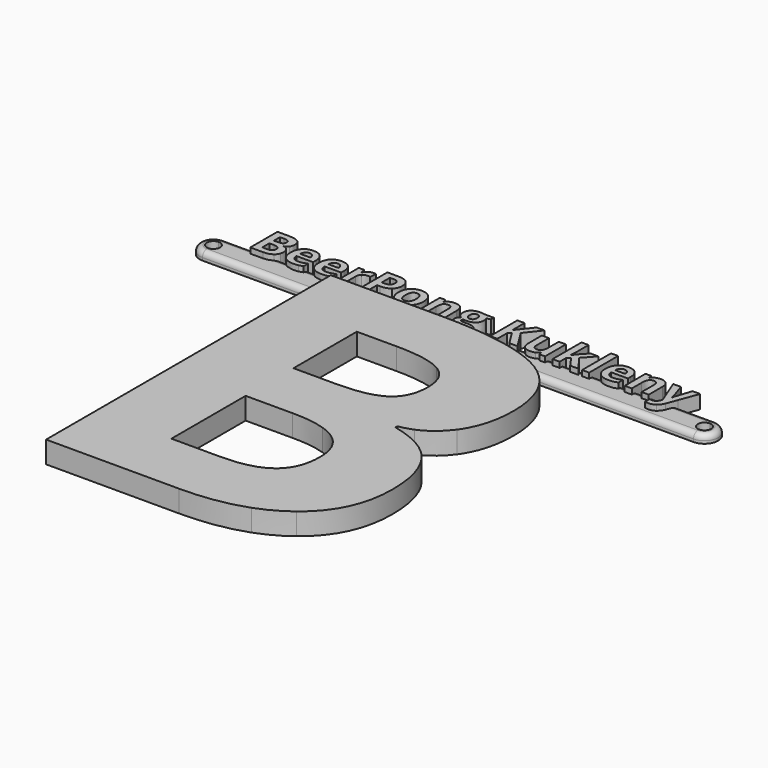
from build123d import *

# Parameters (mm, degrees)
F0_W         = 1.321603928
F0_H         = 1.2847790507
F0_W_2       = 1.2997817785
F1_DEPTH     = 1.5
F2_T1_DEPTH  = 84.4465047724
F2_T3_DEPTH  = 90
F2_T5_DEPTH  = 10.5221227841
F2_T8_ANGLE  = 180
F2_T10_ANGLE = 180
F3_DEPTH     = 2.5
F0_H_2       = 5.3477905074
F4_DEPTH     = 4


# Not quite as in the source:
# - a fillet or chamfer that OpenCascade refuses, or shapes differently, is made with other operations: its cross-section is extruded or revolved along the edge and cut away or added


with BuildPart() as f1:
    # F0 (on Top) → F1 (new body)
    with BuildSketch(Plane.XY):
        with BuildLine():
            ThreePointArc((45, -3.7152209493), (42.5, -1.2152209493), (45, 1.2847790507))
            Line((45, 1.2847790507), (38.1286402838, 1.2847790507))
            Line((38.1286402838, 1.2847790507), (37.4181669394, -0.6096563011))
            add(Edge.make_bspline(
                [(37.4181669394, -0.6096563011), (37.1399345336, -1.3557010366), (36.6264320786, -1.7266775777)],
                knots=[0, 0, 0, 1, 1, 1], degree=2))
            add(Edge.make_bspline(
                [(36.6264320786, -1.7266775777), (36.1129296236, -2.0976541189), (35.4268957992, -2.0976541189)],
                knots=[0, 0, 0, 1, 1, 1], degree=2))
            add(Edge.make_bspline(
                [(35.4268957992, -2.0976541189), (35.0900163666, -2.0976541189), (34.7667757774, -2.0240043644)],
                knots=[0, 0, 0, 1, 1, 1], degree=2))
            Line((34.7667757774, -2.0240043644), (34.7667757774, -0.9929078014))
            add(Edge.make_bspline(
                [(34.7667757774, -0.9929078014), (35.0013638843, -1.0488270595), (35.2782324059, -1.0488270595)],
                knots=[0, 0, 0, 1, 1, 1], degree=2))
            add(Edge.make_bspline(
                [(35.2782324059, -1.0488270595), (35.6232951446, -1.0488270595), (35.8810692853, -0.8374249864)],
                knots=[0, 0, 0, 1, 1, 1], degree=2))
            add(Edge.make_bspline(
                [(35.8810692853, -0.8374249864), (36.1388434261, -0.6260229133), (36.2834151664, -0.2004909984)],
                knots=[0, 0, 0, 1, 1, 1], degree=2))
            Line((36.2834151664, -0.2004909984), (36.3611565739, 0.0340971086))
            Line((36.3611565739, 0.0340971086), (35.8607395847, 1.2847790507))
            Line((35.8607395847, 1.2847790507), (33.8120567376, 1.2847790507))
            Line((33.8120567376, 1.2847790507), (33.8120567376, 0))
            Line((33.8120567376, 0), (32.5122749591, 0))
            Line((32.5122749591, 0), (32.5122749591, 1.2847790507))
            Line((32.5122749591, 1.2847790507), (30.7133115112, 1.2847790507))
            Line((30.7133115112, 1.2847790507), (30.7133115112, 0))
            Line((30.7133115112, 0), (29.4135297327, 0))
            Line((29.4135297327, 0), (29.4135297327, 1.2847790507))
            Line((29.4135297327, 1.2847790507), (25.5323936329, 1.2847790507))
            add(Edge.make_bspline(
                [(25.5323936329, 1.2847790507), (25.5696212292, 1.2367318116), (25.6123840698, 1.1933987998)],
                knots=[0.8606501567, 0.8606501567, 0.8606501567, 1, 1, 1], degree=2))
            add(Edge.make_bspline(
                [(25.6123840698, 1.1933987998), (25.9192580469, 0.8824331697), (26.47299509, 0.8824331697)],
                knots=[0, 0, 0, 1, 1, 1], degree=2))
            add(Edge.make_bspline(
                [(26.47299509, 0.8824331697), (26.9039825423, 0.8824331697), (27.2872340426, 0.9717675941)],
                knots=[0, 0, 0, 1, 1, 1], degree=2))
            add(Edge.make_bspline(
                [(27.2872340426, 0.9717675941), (27.6704855428, 1.0611020185), (28.0878341517, 1.2575013639)],
                knots=[0, 0, 0, 1, 1, 1], degree=2))
            Line((28.0878341517, 1.2575013639), (28.0878341517, 0.250954719))
            add(Edge.make_bspline(
                [(28.0878341517, 0.250954719), (27.746863066, 0.0804691762), (27.3595199127, -0.0027277687)],
                knots=[0, 0, 0, 1, 1, 1], degree=2))
            add(Edge.make_bspline(
                [(27.3595199127, -0.0027277687), (26.9721767594, -0.0859247136), (26.4129841789, -0.0859247136)],
                knots=[0, 0, 0, 1, 1, 1], degree=2))
            add(Edge.make_bspline(
                [(26.4129841789, -0.0859247136), (25.2632296781, -0.0859247136), (24.6153846154, 0.5496453901)],
                knots=[0, 0, 0, 1, 1, 1], degree=2))
            add(Edge.make_bspline(
                [(24.6153846154, 0.5496453901), (24.3031895119, 0.8559252179), (24.1414405386, 1.2847790507)],
                knots=[0, 0, 0, 0.4818977892, 0.4818977892, 0.4818977892], degree=2))
            Line((24.1414405386, 1.2847790507), (22.8927986907, 1.2847790507))
            Line((22.8927986907, 1.2847790507), (22.8927986907, 0))
            Line((22.8927986907, 0), (21.5930169122, 0))
            Line((21.5930169122, 0), (21.5930169122, 1.2847790507))
            Line((21.5930169122, 1.2847790507), (19.9549600985, 1.2847790507))
            Line((19.9549600985, 1.2847790507), (20.9110747409, 0))
            Line((20.9110747409, 0), (19.410801964, 0))
            Line((19.410801964, 0), (18.4980281469, 1.2847790507))
            Line((18.4980281469, 1.2847790507), (17.4795417349, 1.2847790507))
            Line((17.4795417349, 1.2847790507), (17.4795417349, 0))
            Line((17.4795417349, 0), (16.1797599564, 0))
            Line((16.1797599564, 0), (16.1797599564, 1.2847790507))
            Line((16.1797599564, 1.2847790507), (14.8158756137, 1.2847790507))
            Line((14.8158756137, 1.2847790507), (14.8158756137, 0))
            Line((14.8158756137, 0), (13.8188761593, 0))
            Line((13.8188761593, 0), (13.6442989634, 0.6096563011))
            Line((13.6442989634, 0.6096563011), (13.5761047463, 0.6096563011))
            add(Edge.make_bspline(
                [(13.5761047463, 0.6096563011), (13.3674304419, 0.2768685215), (12.9834969995, 0.095471904)],
                knots=[0, 0, 0, 1, 1, 1], degree=2))
            add(Edge.make_bspline(
                [(12.9834969995, 0.095471904), (12.599563557, -0.0859247136), (12.109929078, -0.0859247136)],
                knots=[0, 0, 0, 1, 1, 1], degree=2))
            add(Edge.make_bspline(
                [(12.109929078, -0.0859247136), (11.269776323, -0.0859247136), (10.8435624659, 0.3641571195)],
                knots=[0, 0, 0, 1, 1, 1], degree=2))
            add(Edge.make_bspline(
                [(10.8435624659, 0.3641571195), (10.5171338583, 0.7088657291), (10.4407103458, 1.2847790507)],
                knots=[0, 0, 0, 0.7658798563, 0.7658798563, 0.7658798563], degree=2))
            Line((10.4407103458, 1.2847790507), (8.9512082826, 1.2847790507))
            Line((8.9512082826, 1.2847790507), (9.76132024, 0))
            Line((9.76132024, 0), (8.2610474632, 0))
            Line((8.2610474632, 0), (7.4621484898, 1.2847790507))
            Line((7.4621484898, 1.2847790507), (6.0706492089, 1.2847790507))
            Line((6.0706492089, 1.2847790507), (6.0706492089, 0))
            Line((6.0706492089, 0), (4.749045281, 0))
            Line((4.749045281, 0), (4.749045281, 1.2847790507))
            Line((4.749045281, 1.2847790507), (-1.5938599457, 1.2847790507))
            add(Edge.make_bspline(
                [(-1.5938599457, 1.2847790507), (-1.5943807965, 1.275277922), (-1.5943807965, 1.2656846699)],
                knots=[0.9490306349, 0.9490306349, 0.9490306349, 1, 1, 1], degree=2))
            add(Edge.make_bspline(
                [(-1.5943807965, 1.2656846699), (-1.5943807965, 0.9847244954), (-0.8783415166, 0.9847244954)],
                knots=[0, 0, 0, 1, 1, 1], degree=2))
            Line((-0.8783415166, 0.9847244954), (-0.0681942171, 0.9847244954))
            add(Edge.make_bspline(
                [(-0.0681942171, 0.9847244954), (0.7160392799, 0.9847244954), (1.1272504092, 0.6478450627)],
                knots=[0, 0, 0, 1, 1, 1], degree=2))
            add(Edge.make_bspline(
                [(1.1272504092, 0.6478450627), (1.5384615385, 0.3109656301), (1.5384615385, -0.3409710857)],
                knots=[0, 0, 0, 1, 1, 1], degree=2))
            add(Edge.make_bspline(
                [(1.5384615385, -0.3409710857), (1.5384615385, -0.8967321528), (1.2304984638, -1.2864583333)],
                knots=[0, 0, 0, 0.6647373808, 0.6647373808, 0.6647373808], degree=2))
            Line((1.2304984638, -1.2864583333), (5.4641927083, -1.2864583333))
            Line((5.4641927083, -1.2864583333), (5.7957286846, -2.2259809145))
            add(Edge.make_bspline(
                [(5.7957286846, -2.2259809145), (9.8904888324, -2.7112490445), (12.9853606911, -3.7152209493)],
                knots=[0.3391314157, 0.3391314157, 0.3391314157, 0.7016294547, 0.7016294547, 0.7016294547], degree=2))
            Line((12.9853606911, -3.7152209493), (45, -3.7152209493))
        make_face()
        with BuildLine():
            Line((-45, -3.7152209493), (-23.0418041206, -3.7152209493))
            Line((-23.0418041206, -3.7152209493), (-23.0418041206, -1.7719931678))
            Line((-23.0418041206, -1.7719931678), (-11.6648397723, -1.7719931678))
            Line((-11.6648397723, -1.7719931678), (-11.494140625, -1.2864583333))
            Line((-11.494140625, -1.2864583333), (-3.1010295302, -1.2864583333))
            add(Edge.make_bspline(
                [(-3.1010295302, -1.2864583333), (-3.2092198582, -1.0598434162), (-3.2092198582, -0.7760501909)],
                knots=[0.5466727827, 0.5466727827, 0.5466727827, 1, 1, 1], degree=2))
            add(Edge.make_bspline(
                [(-3.2092198582, -0.7760501909), (-3.2092198582, -0.3450627387), (-2.9405346427, -0.0552373159)],
                knots=[0, 0, 0, 1, 1, 1], degree=2))
            add(Edge.make_bspline(
                [(-2.9405346427, -0.0552373159), (-2.6718494272, 0.2345881069), (-2.1522094926, 0.3587015821)],
                knots=[0, 0, 0, 1, 1, 1], degree=2))
            add(Edge.make_bspline(
                [(-2.1522094926, 0.3587015821), (-2.352700491, 0.4432624113), (-2.5020458265, 0.636933988)],
                knots=[0, 0, 0, 1, 1, 1], degree=2))
            add(Edge.make_bspline(
                [(-2.5020458265, 0.636933988), (-2.651391162, 0.8306055646), (-2.651391162, 1.0488270595)],
                knots=[0, 0, 0, 1, 1, 1], degree=2))
            add(Edge.make_bspline(
                [(-2.651391162, 1.0488270595), (-2.651391162, 1.1769598536), (-2.6166323406, 1.2847790507)],
                knots=[0, 0, 0, 0.4697348232, 0.4697348232, 0.4697348232], degree=2))
            Line((-2.6166323406, 1.2847790507), (-3.8911620295, 1.2847790507))
            Line((-3.8911620295, 1.2847790507), (-3.8911620295, 0))
            Line((-3.8911620295, 0), (-5.190943808, 0))
            Line((-5.190943808, 0), (-5.190943808, 1.2847790507))
            Line((-5.190943808, 1.2847790507), (-6.9899072559, 1.2847790507))
            Line((-6.9899072559, 1.2847790507), (-6.9899072559, 0))
            Line((-6.9899072559, 0), (-8.2896890344, 0))
            Line((-8.2896890344, 0), (-8.2896890344, 1.2847790507))
            Line((-8.2896890344, 1.2847790507), (-9.5424299056, 1.2847790507))
            add(Edge.make_bspline(
                [(-9.5424299056, 1.2847790507), (-9.6949554498, 0.8738335661), (-9.9781778505, 0.5707855974)],
                knots=[0.5385363018, 0.5385363018, 0.5385363018, 1, 1, 1], degree=2))
            add(Edge.make_bspline(
                [(-9.9781778505, 0.5707855974), (-10.5919258047, -0.0859247136), (-11.6871249318, -0.0859247136)],
                knots=[0, 0, 0, 1, 1, 1], degree=2))
            add(Edge.make_bspline(
                [(-11.6871249318, -0.0859247136), (-12.3731587561, -0.0859247136), (-12.8975722859, 0.214811784)],
                knots=[0, 0, 0, 1, 1, 1], degree=2))
            add(Edge.make_bspline(
                [(-12.8975722859, 0.214811784), (-13.4219858156, 0.5155482815), (-13.7029459902, 1.0781505728)],
                knots=[0, 0, 0, 1, 1, 1], degree=2))
            add(Edge.make_bspline(
                [(-13.7029459902, 1.0781505728), (-13.7530512355, 1.1784826781), (-13.794220924, 1.2847790507)],
                knots=[0, 0, 0, 0.1783357566, 0.1783357566, 0.1783357566], degree=2))
            Line((-13.794220924, 1.2847790507), (-17.7523186034, 1.2847790507))
            Line((-17.7523186034, 1.2847790507), (-17.7523186034, 0))
            Line((-17.7523186034, 0), (-19.0739225314, 0))
            Line((-19.0739225314, 0), (-19.0739225314, 1.2847790507))
            Line((-19.0739225314, 1.2847790507), (-21.8398799782, 1.2847790507))
            Line((-21.8398799782, 1.2847790507), (-21.8398799782, 0))
            Line((-21.8398799782, 0), (-23.1396617567, 0))
            Line((-23.1396617567, 0), (-23.1396617567, 1.2847790507))
            Line((-23.1396617567, 1.2847790507), (-27.0207978564, 1.2847790507))
            add(Edge.make_bspline(
                [(-27.0207978564, 1.2847790507), (-26.9835702602, 1.2367318116), (-26.9408074195, 1.1933987998)],
                knots=[0.8606501567, 0.8606501567, 0.8606501567, 1, 1, 1], degree=2))
            add(Edge.make_bspline(
                [(-26.9408074195, 1.1933987998), (-26.6339334424, 0.8824331697), (-26.0801963993, 0.8824331697)],
                knots=[0, 0, 0, 1, 1, 1], degree=2))
            add(Edge.make_bspline(
                [(-26.0801963993, 0.8824331697), (-25.6492089471, 0.8824331697), (-25.2659574468, 0.9717675941)],
                knots=[0, 0, 0, 1, 1, 1], degree=2))
            add(Edge.make_bspline(
                [(-25.2659574468, 0.9717675941), (-24.8827059465, 1.0611020185), (-24.4653573377, 1.2575013639)],
                knots=[0, 0, 0, 1, 1, 1], degree=2))
            Line((-24.4653573377, 1.2575013639), (-24.4653573377, 0.250954719))
            add(Edge.make_bspline(
                [(-24.4653573377, 0.250954719), (-24.8063284233, 0.0804691762), (-25.1936715767, -0.0027277687)],
                knots=[0, 0, 0, 1, 1, 1], degree=2))
            add(Edge.make_bspline(
                [(-25.1936715767, -0.0027277687), (-25.58101473, -0.0859247136), (-26.1402073104, -0.0859247136)],
                knots=[0, 0, 0, 1, 1, 1], degree=2))
            add(Edge.make_bspline(
                [(-26.1402073104, -0.0859247136), (-27.2899618112, -0.0859247136), (-27.937806874, 0.5496453901)],
                knots=[0, 0, 0, 1, 1, 1], degree=2))
            add(Edge.make_bspline(
                [(-27.937806874, 0.5496453901), (-28.2500019775, 0.8559252179), (-28.4117509508, 1.2847790507)],
                knots=[0, 0, 0, 0.4818977892, 0.4818977892, 0.4818977892], degree=2))
            Line((-28.4117509508, 1.2847790507), (-32.1776445558, 1.2847790507))
            add(Edge.make_bspline(
                [(-32.1776445558, 1.2847790507), (-32.1404169596, 1.2367318116), (-32.0976541189, 1.1933987998)],
                knots=[0.8606501567, 0.8606501567, 0.8606501567, 1, 1, 1], degree=2))
            add(Edge.make_bspline(
                [(-32.0976541189, 1.1933987998), (-31.7907801418, 0.8824331697), (-31.2370430987, 0.8824331697)],
                knots=[0, 0, 0, 1, 1, 1], degree=2))
            add(Edge.make_bspline(
                [(-31.2370430987, 0.8824331697), (-30.8060556465, 0.8824331697), (-30.4228041462, 0.9717675941)],
                knots=[0, 0, 0, 1, 1, 1], degree=2))
            add(Edge.make_bspline(
                [(-30.4228041462, 0.9717675941), (-30.0395526459, 1.0611020185), (-29.6222040371, 1.2575013639)],
                knots=[0, 0, 0, 1, 1, 1], degree=2))
            Line((-29.6222040371, 1.2575013639), (-29.6222040371, 0.250954719))
            add(Edge.make_bspline(
                [(-29.6222040371, 0.250954719), (-29.9631751227, 0.0804691762), (-30.3505182761, -0.0027277687)],
                knots=[0, 0, 0, 1, 1, 1], degree=2))
            add(Edge.make_bspline(
                [(-30.3505182761, -0.0027277687), (-30.7378614294, -0.0859247136), (-31.2970540098, -0.0859247136)],
                knots=[0, 0, 0, 1, 1, 1], degree=2))
            add(Edge.make_bspline(
                [(-31.2970540098, -0.0859247136), (-32.4468085106, -0.0859247136), (-33.0946535734, 0.5496453901)],
                knots=[0, 0, 0, 1, 1, 1], degree=2))
            add(Edge.make_bspline(
                [(-33.0946535734, 0.5496453901), (-33.4068486769, 0.8559252179), (-33.5685976502, 1.2847790507)],
                knots=[0, 0, 0, 0.4818977892, 0.4818977892, 0.4818977892], degree=2))
            Line((-33.5685976502, 1.2847790507), (-34.6622310865, 1.2847790507))
            add(Edge.make_bspline(
                [(-34.6622310865, 1.2847790507), (-34.7986215537, 0.7969904531), (-35.2114020731, 0.4773595199)],
                knots=[0.3304188566, 0.3304188566, 0.3304188566, 1, 1, 1], degree=2))
            add(Edge.make_bspline(
                [(-35.2114020731, 0.4773595199), (-35.827877796, 0), (-36.8848881615, 0)],
                knots=[0, 0, 0, 1, 1, 1], degree=2))
            Line((-36.8848881615, 0), (-39.215766503, 0))
            Line((-39.215766503, 0), (-39.215766503, 1.2847790507))
            Line((-39.215766503, 1.2847790507), (-45, 1.2847790507))
            ThreePointArc((-45, 1.2847790507), (-43.232233047, 0.5525460037), (-42.5, -1.2152209493))
            ThreePointArc((-42.5, -1.2152209493), (-43.232233047, -2.9829879022), (-45, -3.7152209493))
        make_face()
        with BuildLine():
            Line((-12.3480190251, -3.7152209493), (6.3212473455, -3.7152209493))
            Line((6.3212473455, -3.7152209493), (5.7957286846, -2.2259809145))
            add(Edge.make_bspline(
                [(0.4791361693, -1.8288129303), (3.3201638221, -1.9326028684), (5.7957286846, -2.2259809145)],
                knots=[0.1199763552, 0.1199763552, 0.1199763552, 0.3391314157, 0.3391314157, 0.3391314157], degree=2))
            add(Edge.make_bspline(
                [(0.4791361693, -1.8288129303), (-0.1628467181, -2.0976541189), (-1.1593016912, -2.0976541189)],
                knots=[0.2357732361, 0.2357732361, 0.2357732361, 1, 1, 1], degree=2))
            add(Edge.make_bspline(
                [(-1.1593016912, -2.0976541189), (-2.1239952165, -2.0976541189), (-2.6481485619, -1.7720374642)],
                knots=[0, 0, 0, 0.9675968437, 0.9675968437, 0.9675968437], degree=2))
            add(Edge.make_bspline(
                [(-2.7410324604, -1.7719931678), (-2.6945478168, -1.7719931678), (-2.6481485619, -1.7720374642)],
                knots=[0, 0, 0, 0.003349888, 0.003349888, 0.003349888], degree=2))
            Line((-2.7410324604, -1.7719931678), (-11.6648397723, -1.7719931678))
            Line((-11.6648397723, -1.7719931678), (-12.3480190251, -3.7152209493))
        make_face()
        Polygon((-23.0418041206, -3.7152209493), (-12.3480190251, -3.7152209493), (-11.6648397723, -1.7719931678), (-23.0418041206, -1.7719931678), align=None)
        with BuildLine():
            Line((-3.1010295302, -1.2864583333), (1.2304984638, -1.2864583333))
            add(Edge.make_bspline(
                [(1.5384615385, -0.3409710857), (1.5384615385, -0.8967321528), (1.2304984638, -1.2864583333)],
                knots=[0, 0, 0, 0.6647373808, 0.6647373808, 0.6647373808], degree=2))
            add(Edge.make_bspline(
                [(1.1272504092, 0.6478450627), (1.5384615385, 0.3109656301), (1.5384615385, -0.3409710857)],
                knots=[0, 0, 0, 1, 1, 1], degree=2))
            add(Edge.make_bspline(
                [(-0.0681942171, 0.9847244954), (0.7160392799, 0.9847244954), (1.1272504092, 0.6478450627)],
                knots=[0, 0, 0, 1, 1, 1], degree=2))
            Line((-0.0681942171, 0.9847244954), (-0.8783415166, 0.9847244954))
            add(Edge.make_bspline(
                [(-1.5943807965, 1.2656846699), (-1.5943807965, 0.9847244954), (-0.8783415166, 0.9847244954)],
                knots=[0, 0, 0, 1, 1, 1], degree=2))
            add(Edge.make_bspline(
                [(-1.5938599457, 1.2847790507), (-1.5943807965, 1.275277922), (-1.5943807965, 1.2656846699)],
                knots=[0.9490306349, 0.9490306349, 0.9490306349, 1, 1, 1], degree=2))
            Line((-1.5938599457, 1.2847790507), (-2.6166323406, 1.2847790507))
            add(Edge.make_bspline(
                [(-2.651391162, 1.0488270595), (-2.651391162, 1.1769598536), (-2.6166323406, 1.2847790507)],
                knots=[0, 0, 0, 0.4697348232, 0.4697348232, 0.4697348232], degree=2))
            add(Edge.make_bspline(
                [(-2.5020458265, 0.636933988), (-2.651391162, 0.8306055646), (-2.651391162, 1.0488270595)],
                knots=[0, 0, 0, 1, 1, 1], degree=2))
            add(Edge.make_bspline(
                [(-2.1522094926, 0.3587015821), (-2.352700491, 0.4432624113), (-2.5020458265, 0.636933988)],
                knots=[0, 0, 0, 1, 1, 1], degree=2))
            add(Edge.make_bspline(
                [(-2.9405346427, -0.0552373159), (-2.6718494272, 0.2345881069), (-2.1522094926, 0.3587015821)],
                knots=[0, 0, 0, 1, 1, 1], degree=2))
            add(Edge.make_bspline(
                [(-3.2092198582, -0.7760501909), (-3.2092198582, -0.3450627387), (-2.9405346427, -0.0552373159)],
                knots=[0, 0, 0, 1, 1, 1], degree=2))
            add(Edge.make_bspline(
                [(-3.1010295302, -1.2864583333), (-3.2092198582, -1.0598434162), (-3.2092198582, -0.7760501909)],
                knots=[0.5466727827, 0.5466727827, 0.5466727827, 1, 1, 1], degree=2))
        make_face()
        with BuildLine():
            add(Edge.make_bspline(
                [(-2.0840152755, -0.6737588652), (-2.0840152755, -0.9424440807), (-1.8262411348, -1.0958810693)],
                knots=[0, 0, 0, 1, 1, 1], degree=2))
            add(Edge.make_bspline(
                [(-1.843289689, -0.2284506274), (-2.0840152755, -0.3968903437), (-2.0840152755, -0.6737588652)],
                knots=[0, 0, 0, 1, 1, 1], degree=2))
            add(Edge.make_bspline(
                [(-1.2452264048, -0.0600109111), (-1.6025641026, -0.0600109111), (-1.843289689, -0.2284506274)],
                knots=[0, 0, 0, 1, 1, 1], degree=2))
            Line((-1.2452264048, -0.0600109111), (-0.5714675396, -0.0600109111))
            add(Edge.make_bspline(
                [(0.1534369885, -0.1623022368), (-0.0804691762, -0.0600109111), (-0.5714675396, -0.0600109111)],
                knots=[0, 0, 0, 1, 1, 1], degree=2))
            add(Edge.make_bspline(
                [(0.3873431533, -0.533278778), (0.3873431533, -0.2645935625), (0.1534369885, -0.1623022368)],
                knots=[0, 0, 0, 1, 1, 1], degree=2))
            add(Edge.make_bspline(
                [(-0.0088652482, -1.0570103655), (0.3873431533, -0.8647026732), (0.3873431533, -0.533278778)],
                knots=[0, 0, 0, 1, 1, 1], degree=2))
            add(Edge.make_bspline(
                [(-1.1033824332, -1.2493180578), (-0.4050736498, -1.2493180578), (-0.0088652482, -1.0570103655)],
                knots=[0, 0, 0, 1, 1, 1], degree=2))
            add(Edge.make_bspline(
                [(-1.8262411348, -1.0958810693), (-1.568466994, -1.2493180578), (-1.1033824332, -1.2493180578)],
                knots=[0, 0, 0, 1, 1, 1], degree=2))
        make_face(mode=Mode.SUBTRACT)
        with BuildLine():
            Line((-45, -2.4304418985), (-45, -3.7152209493))
            ThreePointArc((-45, -3.7152209493), (-43.232233047, -2.9829879022), (-42.5, -1.2152209493))
            ThreePointArc((-42.5, -1.2152209493), (-43.232233047, 0.5525460037), (-45, 1.2847790507))
            Line((-45, 1.2847790507), (-45, 0))
            ThreePointArc((-45, 0), (-44.1407090261, -0.3559299754), (-43.7847790507, -1.2152209493))
            ThreePointArc((-43.7847790507, -1.2152209493), (-44.1407090261, -2.0745119231), (-45, -2.4304418985))
        make_face()
        with BuildLine():
            ThreePointArc((-45, 1.2847790507), (-47.5, -1.2152209493), (-45, -3.7152209493))
            Line((-45, -3.7152209493), (-45, -2.4304418985))
            ThreePointArc((-45, -2.4304418985), (-46.2152209493, -1.2152209493), (-45, 0))
            Line((-45, 0), (-45, 1.2847790507))
        make_face()
        with BuildLine():
            Line((45, 0), (45, 1.2847790507))
            ThreePointArc((45, 1.2847790507), (42.5, -1.2152209493), (45, -3.7152209493))
            Line((45, -3.7152209493), (45, -2.4304418985))
            ThreePointArc((45, -2.4304418985), (43.7847790507, -1.2152209493), (45, 0))
        make_face()
        with BuildLine():
            ThreePointArc((47.5, -1.2152209493), (46.767766953, 0.5525460037), (45, 1.2847790507))
            Line((45, 1.2847790507), (45, 0))
            ThreePointArc((45, 0), (45.8592909739, -0.3559299754), (46.2152209493, -1.2152209493))
            ThreePointArc((46.2152209493, -1.2152209493), (45.8592909739, -2.0745119231), (45, -2.4304418985))
            Line((45, -2.4304418985), (45, -3.7152209493))
            ThreePointArc((45, -3.7152209493), (46.767766953, -2.9829879022), (47.5, -1.2152209493))
        make_face()
        with BuildLine():
            Line((6.3212473455, -3.7152209493), (12.9853606911, -3.7152209493))
            add(Edge.make_bspline(
                [(5.7957286846, -2.2259809145), (9.8904888324, -2.7112490445), (12.9853606911, -3.7152209493)],
                knots=[0.3391314157, 0.3391314157, 0.3391314157, 0.7016294547, 0.7016294547, 0.7016294547], degree=2))
            Line((5.7957286846, -2.2259809145), (6.3212473455, -3.7152209493))
        make_face()
        with BuildLine():
            Line((37.4181669394, -0.6096563011), (38.1286402838, 1.2847790507))
            Line((38.1286402838, 1.2847790507), (36.9778772159, 1.2847790507))
            add(Edge.make_bspline(
                [(36.9749045281, 1.2575013639), (36.9763473032, 1.2711652924), (36.9778772159, 1.2847790507)],
                knots=[0, 0, 0, 0.0311130198, 0.0311130198, 0.0311130198], degree=2))
            Line((36.9749045281, 1.2575013639), (36.9489907256, 1.2575013639))
            add(Edge.make_bspline(
                [(36.9465047724, 1.2847790507), (36.947778043, 1.2711929414), (36.9489907256, 1.2575013639)],
                knots=[0.9713181011, 0.9713181011, 0.9713181011, 1, 1, 1], degree=2))
            Line((36.9465047724, 1.2847790507), (35.8607395847, 1.2847790507))
            Line((35.8607395847, 1.2847790507), (36.3611565739, 0.0340971086))
            Line((36.3611565739, 0.0340971086), (36.2834151664, -0.2004909984))
            add(Edge.make_bspline(
                [(35.8810692853, -0.8374249864), (36.1388434261, -0.6260229133), (36.2834151664, -0.2004909984)],
                knots=[0, 0, 0, 1, 1, 1], degree=2))
            add(Edge.make_bspline(
                [(35.2782324059, -1.0488270595), (35.6232951446, -1.0488270595), (35.8810692853, -0.8374249864)],
                knots=[0, 0, 0, 1, 1, 1], degree=2))
            add(Edge.make_bspline(
                [(34.7667757774, -0.9929078014), (35.0013638843, -1.0488270595), (35.2782324059, -1.0488270595)],
                knots=[0, 0, 0, 1, 1, 1], degree=2))
            Line((34.7667757774, -0.9929078014), (34.7667757774, -2.0240043644))
            add(Edge.make_bspline(
                [(35.4268957992, -2.0976541189), (35.0900163666, -2.0976541189), (34.7667757774, -2.0240043644)],
                knots=[0, 0, 0, 1, 1, 1], degree=2))
            add(Edge.make_bspline(
                [(36.6264320786, -1.7266775777), (36.1129296236, -2.0976541189), (35.4268957992, -2.0976541189)],
                knots=[0, 0, 0, 1, 1, 1], degree=2))
            add(Edge.make_bspline(
                [(37.4181669394, -0.6096563011), (37.1399345336, -1.3557010366), (36.6264320786, -1.7266775777)],
                knots=[0, 0, 0, 1, 1, 1], degree=2))
        make_face()
        with BuildLine():
            Line((-37.894162575, 1.2847790507), (-39.215766503, 1.2847790507))
            Line((-39.215766503, 1.2847790507), (-39.215766503, 0))
            Line((-39.215766503, 0), (-36.8848881615, 0))
            add(Edge.make_bspline(
                [(-35.2114020731, 0.4773595199), (-35.827877796, 0), (-36.8848881615, 0)],
                knots=[0, 0, 0, 1, 1, 1], degree=2))
            add(Edge.make_bspline(
                [(-34.6622310865, 1.2847790507), (-34.7986215537, 0.7969904531), (-35.2114020731, 0.4773595199)],
                knots=[0.3304188566, 0.3304188566, 0.3304188566, 1, 1, 1], degree=2))
            Line((-34.6622310865, 1.2847790507), (-36.2475892447, 1.2847790507))
            add(Edge.make_bspline(
                [(-37.0335515548, 1.0911074741), (-36.5079749903, 1.0911074741), (-36.2475892447, 1.2847790507)],
                knots=[0, 0, 0, 0.9633818429, 0.9633818429, 0.9633818429], degree=2))
            Line((-37.0335515548, 1.0911074741), (-37.894162575, 1.0911074741))
            Line((-37.894162575, 1.0911074741), (-37.894162575, 1.2847790507))
        make_face()
        with BuildLine():
            Line((11.8532622832, 1.2847790507), (10.4407103458, 1.2847790507))
            add(Edge.make_bspline(
                [(10.8435624659, 0.3641571195), (10.5171338583, 0.7088657291), (10.4407103458, 1.2847790507)],
                knots=[0, 0, 0, 0.7658798563, 0.7658798563, 0.7658798563], degree=2))
            add(Edge.make_bspline(
                [(12.109929078, -0.0859247136), (11.269776323, -0.0859247136), (10.8435624659, 0.3641571195)],
                knots=[0, 0, 0, 1, 1, 1], degree=2))
            add(Edge.make_bspline(
                [(12.9834969995, 0.095471904), (12.599563557, -0.0859247136), (12.109929078, -0.0859247136)],
                knots=[0, 0, 0, 1, 1, 1], degree=2))
            add(Edge.make_bspline(
                [(13.5761047463, 0.6096563011), (13.3674304419, 0.2768685215), (12.9834969995, 0.095471904)],
                knots=[0, 0, 0, 1, 1, 1], degree=2))
            Line((13.5761047463, 0.6096563011), (13.6442989634, 0.6096563011))
            Line((13.6442989634, 0.6096563011), (13.8188761593, 0))
            Line((13.8188761593, 0), (14.8158756137, 0))
            Line((14.8158756137, 0), (14.8158756137, 1.2847790507))
            Line((14.8158756137, 1.2847790507), (13.2523525736, 1.2847790507))
            add(Edge.make_bspline(
                [(12.4849972722, 0.9506273868), (13.0075919068, 0.9506273868), (13.2523525736, 1.2847790507)],
                knots=[0, 0, 0, 0.9579159651, 0.9579159651, 0.9579159651], degree=2))
            add(Edge.make_bspline(
                [(11.9005728314, 1.2084015276), (12.0840152755, 0.9506273868), (12.4849972722, 0.9506273868)],
                knots=[0, 0, 0, 1, 1, 1], degree=2))
            add(Edge.make_bspline(
                [(11.8532622832, 1.2847790507), (11.8751568652, 1.2441161567), (11.9005728314, 1.2084015276)],
                knots=[0.8614499149, 0.8614499149, 0.8614499149, 1, 1, 1], degree=2))
        make_face()
        with BuildLine():
            Line((-11.494140625, -1.2864583333), (-11.6648397723, -1.7719931678))
            Line((-11.6648397723, -1.7719931678), (-2.7410324604, -1.7719931678))
            add(Edge.make_bspline(
                [(-2.7410324604, -1.7719931678), (-2.6945478168, -1.7719931678), (-2.6481485619, -1.7720374642)],
                knots=[0, 0, 0, 0.003349888, 0.003349888, 0.003349888], degree=2))
            add(Edge.make_bspline(
                [(-2.6481485619, -1.7720374642), (-2.6657015571, -1.7611331217), (-2.6827605019, -1.7498636116)],
                knots=[0.9675968437, 0.9675968437, 0.9675968437, 1, 1, 1], degree=2))
            add(Edge.make_bspline(
                [(-2.6827605019, -1.7498636116), (-2.9705615032, -1.5597360071), (-3.1010295302, -1.2864583333)],
                knots=[0, 0, 0, 0.5466727827, 0.5466727827, 0.5466727827], degree=2))
            Line((-3.1010295302, -1.2864583333), (-11.494140625, -1.2864583333))
        make_face()
        with BuildLine():
            add(Edge.make_bspline(
                [(-9.5424299056, 1.2847790507), (-9.6949554498, 0.8738335661), (-9.9781778505, 0.5707855974)],
                knots=[0.5385363018, 0.5385363018, 0.5385363018, 1, 1, 1], degree=2))
            Line((-9.5424299056, 1.2847790507), (-10.9447816586, 1.2847790507))
            add(Edge.make_bspline(
                [(-11.6707583197, 0.9588106929), (-11.1750366616, 0.9588106929), (-10.9447816586, 1.2847790507)],
                knots=[0, 0, 0, 0.9514741354, 0.9514741354, 0.9514741354], degree=2))
            add(Edge.make_bspline(
                [(-12.4024478859, 1.2847790507), (-12.16766571, 0.9588106929), (-11.6707583197, 0.9588106929)],
                knots=[0.0512174517, 0.0512174517, 0.0512174517, 1, 1, 1], degree=2))
            Line((-12.4024478859, 1.2847790507), (-13.794220924, 1.2847790507))
            add(Edge.make_bspline(
                [(-13.7029459902, 1.0781505728), (-13.7530512355, 1.1784826781), (-13.794220924, 1.2847790507)],
                knots=[0, 0, 0, 0.1783357566, 0.1783357566, 0.1783357566], degree=2))
            add(Edge.make_bspline(
                [(-12.8975722859, 0.214811784), (-13.4219858156, 0.5155482815), (-13.7029459902, 1.0781505728)],
                knots=[0, 0, 0, 1, 1, 1], degree=2))
            add(Edge.make_bspline(
                [(-11.6871249318, -0.0859247136), (-12.3731587561, -0.0859247136), (-12.8975722859, 0.214811784)],
                knots=[0, 0, 0, 1, 1, 1], degree=2))
            add(Edge.make_bspline(
                [(-9.9781778505, 0.5707855974), (-10.5919258047, -0.0859247136), (-11.6871249318, -0.0859247136)],
                knots=[0, 0, 0, 1, 1, 1], degree=2))
        make_face()
        with BuildLine():
            Line((-32.1776445558, 1.2847790507), (-33.5685976502, 1.2847790507))
            add(Edge.make_bspline(
                [(-33.0946535734, 0.5496453901), (-33.4068486769, 0.8559252179), (-33.5685976502, 1.2847790507)],
                knots=[0, 0, 0, 0.4818977892, 0.4818977892, 0.4818977892], degree=2))
            add(Edge.make_bspline(
                [(-31.2970540098, -0.0859247136), (-32.4468085106, -0.0859247136), (-33.0946535734, 0.5496453901)],
                knots=[0, 0, 0, 1, 1, 1], degree=2))
            add(Edge.make_bspline(
                [(-30.3505182761, -0.0027277687), (-30.7378614294, -0.0859247136), (-31.2970540098, -0.0859247136)],
                knots=[0, 0, 0, 1, 1, 1], degree=2))
            add(Edge.make_bspline(
                [(-29.6222040371, 0.250954719), (-29.9631751227, 0.0804691762), (-30.3505182761, -0.0027277687)],
                knots=[0, 0, 0, 1, 1, 1], degree=2))
            Line((-29.6222040371, 0.250954719), (-29.6222040371, 1.2575013639))
            add(Edge.make_bspline(
                [(-30.4228041462, 0.9717675941), (-30.0395526459, 1.0611020185), (-29.6222040371, 1.2575013639)],
                knots=[0, 0, 0, 1, 1, 1], degree=2))
            add(Edge.make_bspline(
                [(-31.2370430987, 0.8824331697), (-30.8060556465, 0.8824331697), (-30.4228041462, 0.9717675941)],
                knots=[0, 0, 0, 1, 1, 1], degree=2))
            add(Edge.make_bspline(
                [(-32.0976541189, 1.1933987998), (-31.7907801418, 0.8824331697), (-31.2370430987, 0.8824331697)],
                knots=[0, 0, 0, 1, 1, 1], degree=2))
            add(Edge.make_bspline(
                [(-32.1776445558, 1.2847790507), (-32.1404169596, 1.2367318116), (-32.0976541189, 1.1933987998)],
                knots=[0.8606501567, 0.8606501567, 0.8606501567, 1, 1, 1], degree=2))
        make_face()
        with BuildLine():
            Line((-27.0207978564, 1.2847790507), (-28.4117509508, 1.2847790507))
            add(Edge.make_bspline(
                [(-27.937806874, 0.5496453901), (-28.2500019775, 0.8559252179), (-28.4117509508, 1.2847790507)],
                knots=[0, 0, 0, 0.4818977892, 0.4818977892, 0.4818977892], degree=2))
            add(Edge.make_bspline(
                [(-26.1402073104, -0.0859247136), (-27.2899618112, -0.0859247136), (-27.937806874, 0.5496453901)],
                knots=[0, 0, 0, 1, 1, 1], degree=2))
            add(Edge.make_bspline(
                [(-25.1936715767, -0.0027277687), (-25.58101473, -0.0859247136), (-26.1402073104, -0.0859247136)],
                knots=[0, 0, 0, 1, 1, 1], degree=2))
            add(Edge.make_bspline(
                [(-24.4653573377, 0.250954719), (-24.8063284233, 0.0804691762), (-25.1936715767, -0.0027277687)],
                knots=[0, 0, 0, 1, 1, 1], degree=2))
            Line((-24.4653573377, 0.250954719), (-24.4653573377, 1.2575013639))
            add(Edge.make_bspline(
                [(-25.2659574468, 0.9717675941), (-24.8827059465, 1.0611020185), (-24.4653573377, 1.2575013639)],
                knots=[0, 0, 0, 1, 1, 1], degree=2))
            add(Edge.make_bspline(
                [(-26.0801963993, 0.8824331697), (-25.6492089471, 0.8824331697), (-25.2659574468, 0.9717675941)],
                knots=[0, 0, 0, 1, 1, 1], degree=2))
            add(Edge.make_bspline(
                [(-26.9408074195, 1.1933987998), (-26.6339334424, 0.8824331697), (-26.0801963993, 0.8824331697)],
                knots=[0, 0, 0, 1, 1, 1], degree=2))
            add(Edge.make_bspline(
                [(-27.0207978564, 1.2847790507), (-26.9835702602, 1.2367318116), (-26.9408074195, 1.1933987998)],
                knots=[0.8606501567, 0.8606501567, 0.8606501567, 1, 1, 1], degree=2))
        make_face()
        with BuildLine():
            add(Edge.make_bspline(
                [(25.5323936329, 1.2847790507), (25.5696212292, 1.2367318116), (25.6123840698, 1.1933987998)],
                knots=[0.8606501567, 0.8606501567, 0.8606501567, 1, 1, 1], degree=2))
            Line((25.5323936329, 1.2847790507), (24.1414405386, 1.2847790507))
            add(Edge.make_bspline(
                [(24.6153846154, 0.5496453901), (24.3031895119, 0.8559252179), (24.1414405386, 1.2847790507)],
                knots=[0, 0, 0, 0.4818977892, 0.4818977892, 0.4818977892], degree=2))
            add(Edge.make_bspline(
                [(26.4129841789, -0.0859247136), (25.2632296781, -0.0859247136), (24.6153846154, 0.5496453901)],
                knots=[0, 0, 0, 1, 1, 1], degree=2))
            add(Edge.make_bspline(
                [(27.3595199127, -0.0027277687), (26.9721767594, -0.0859247136), (26.4129841789, -0.0859247136)],
                knots=[0, 0, 0, 1, 1, 1], degree=2))
            add(Edge.make_bspline(
                [(28.0878341517, 0.250954719), (27.746863066, 0.0804691762), (27.3595199127, -0.0027277687)],
                knots=[0, 0, 0, 1, 1, 1], degree=2))
            Line((28.0878341517, 0.250954719), (28.0878341517, 1.2575013639))
            add(Edge.make_bspline(
                [(27.2872340426, 0.9717675941), (27.6704855428, 1.0611020185), (28.0878341517, 1.2575013639)],
                knots=[0, 0, 0, 1, 1, 1], degree=2))
            add(Edge.make_bspline(
                [(26.47299509, 0.8824331697), (26.9039825423, 0.8824331697), (27.2872340426, 0.9717675941)],
                knots=[0, 0, 0, 1, 1, 1], degree=2))
            add(Edge.make_bspline(
                [(25.6123840698, 1.1933987998), (25.9192580469, 0.8824331697), (26.47299509, 0.8824331697)],
                knots=[0, 0, 0, 1, 1, 1], degree=2))
        make_face()
        with BuildLine():
            add(Edge.make_bspline(
                [(0.4791361693, -1.8288129303), (3.3201638221, -1.9326028684), (5.7957286846, -2.2259809145)],
                knots=[0.1199763552, 0.1199763552, 0.1199763552, 0.3391314157, 0.3391314157, 0.3391314157], degree=2))
            Line((5.7957286846, -2.2259809145), (5.4641927083, -1.2864583333))
            Line((5.4641927083, -1.2864583333), (1.2304984638, -1.2864583333))
            add(Edge.make_bspline(
                [(1.2304984638, -1.2864583333), (1.0751762117, -1.4830180933), (0.8415166394, -1.6373431533)],
                knots=[0.6647373808, 0.6647373808, 0.6647373808, 1, 1, 1], degree=2))
            add(Edge.make_bspline(
                [(0.8415166394, -1.6373431533), (0.6771956852, -1.7458721593), (0.4791361693, -1.8288129303)],
                knots=[0, 0, 0, 0.2357732361, 0.2357732361, 0.2357732361], degree=2))
        make_face()
        with BuildLine():
            add(Edge.make_bspline(
                [(-1.843289689, -0.2284506274), (-2.0840152755, -0.3968903437), (-2.0840152755, -0.6737588652)],
                knots=[0, 0, 0, 1, 1, 1], degree=2))
            add(Edge.make_bspline(
                [(-2.0840152755, -0.6737588652), (-2.0840152755, -0.9424440807), (-1.8262411348, -1.0958810693)],
                knots=[0, 0, 0, 1, 1, 1], degree=2))
            add(Edge.make_bspline(
                [(-1.8262411348, -1.0958810693), (-1.568466994, -1.2493180578), (-1.1033824332, -1.2493180578)],
                knots=[0, 0, 0, 1, 1, 1], degree=2))
            add(Edge.make_bspline(
                [(-1.1033824332, -1.2493180578), (-0.4050736498, -1.2493180578), (-0.0088652482, -1.0570103655)],
                knots=[0, 0, 0, 1, 1, 1], degree=2))
            add(Edge.make_bspline(
                [(-0.0088652482, -1.0570103655), (0.3873431533, -0.8647026732), (0.3873431533, -0.533278778)],
                knots=[0, 0, 0, 1, 1, 1], degree=2))
            add(Edge.make_bspline(
                [(0.3873431533, -0.533278778), (0.3873431533, -0.2645935625), (0.1534369885, -0.1623022368)],
                knots=[0, 0, 0, 1, 1, 1], degree=2))
            add(Edge.make_bspline(
                [(0.1534369885, -0.1623022368), (-0.0804691762, -0.0600109111), (-0.5714675396, -0.0600109111)],
                knots=[0, 0, 0, 1, 1, 1], degree=2))
            Line((-0.5714675396, -0.0600109111), (-1.2452264048, -0.0600109111))
            add(Edge.make_bspline(
                [(-1.2452264048, -0.0600109111), (-1.6025641026, -0.0600109111), (-1.843289689, -0.2284506274)],
                knots=[0, 0, 0, 1, 1, 1], degree=2))
        make_face()
        with BuildLine():
            add(Edge.make_bspline(
                [(-2.6481485619, -1.7720374642), (-1.0327569053, -1.7735796457), (0.4791361693, -1.8288129303)],
                knots=[0.003349888, 0.003349888, 0.003349888, 0.1199763552, 0.1199763552, 0.1199763552], degree=2))
            add(Edge.make_bspline(
                [(0.8415166394, -1.6373431533), (0.6771956852, -1.7458721593), (0.4791361693, -1.8288129303)],
                knots=[0, 0, 0, 0.2357732361, 0.2357732361, 0.2357732361], degree=2))
            add(Edge.make_bspline(
                [(1.2304984638, -1.2864583333), (1.0751762117, -1.4830180933), (0.8415166394, -1.6373431533)],
                knots=[0.6647373808, 0.6647373808, 0.6647373808, 1, 1, 1], degree=2))
            Line((1.2304984638, -1.2864583333), (-3.1010295302, -1.2864583333))
            add(Edge.make_bspline(
                [(-2.6827605019, -1.7498636116), (-2.9705615032, -1.5597360071), (-3.1010295302, -1.2864583333)],
                knots=[0, 0, 0, 0.5466727827, 0.5466727827, 0.5466727827], degree=2))
            add(Edge.make_bspline(
                [(-2.6481485619, -1.7720374642), (-2.6657015571, -1.7611331217), (-2.6827605019, -1.7498636116)],
                knots=[0.9675968437, 0.9675968437, 0.9675968437, 1, 1, 1], degree=2))
        make_face()
        Polygon((8.9512082826, 1.2847790507), (7.4621484898, 1.2847790507), (8.2610474632, 0), (9.76132024, 0), align=None)
        Polygon((20.9110747409, 0), (19.9549600985, 1.2847790507), (18.4980281469, 1.2847790507), (19.410801964, 0), align=None)
        with Locations((-18.4131205674, 0.6423895254)):
            Rectangle(F0_W, F0_H)
        with Locations((5.409847245, 0.6423895254)):
            Rectangle(F0_W, F0_H)
        with Locations((-22.4897708674, 0.6423895254)):
            Rectangle(F0_W_2, F0_H)
        with Locations((16.8296508456, 0.6423895254)):
            Rectangle(F0_W_2, F0_H)
        with Locations((22.2429078014, 0.6423895254)):
            Rectangle(F0_W_2, F0_H)
        with Locations((30.0634206219, 0.6423895254)):
            Rectangle(F0_W_2, F0_H)
        with Locations((33.1621658483, 0.6423895254)):
            Rectangle(F0_W_2, F0_H)
        with Locations((-7.6397981451, 0.6423895254)):
            Rectangle(F0_W_2, F0_H)
        with Locations((-4.5410529187, 0.6423895254)):
            Rectangle(F0_W_2, F0_H)
        with BuildLine():
            add(Edge.make_bspline(
                [(0.4791361693, -1.8288129303), (-0.1628467181, -2.0976541189), (-1.1593016912, -2.0976541189)],
                knots=[0.2357732361, 0.2357732361, 0.2357732361, 1, 1, 1], degree=2))
            add(Edge.make_bspline(
                [(-2.6481485619, -1.7720374642), (-1.0327569053, -1.7735796457), (0.4791361693, -1.8288129303)],
                knots=[0.003349888, 0.003349888, 0.003349888, 0.1199763552, 0.1199763552, 0.1199763552], degree=2))
            add(Edge.make_bspline(
                [(-1.1593016912, -2.0976541189), (-2.1239952165, -2.0976541189), (-2.6481485619, -1.7720374642)],
                knots=[0, 0, 0, 0.9675968437, 0.9675968437, 0.9675968437], degree=2))
        make_face()
        with BuildLine():
            add(Edge.make_bspline(
                [(-11.6707583197, 0.9588106929), (-11.1750366616, 0.9588106929), (-10.9447816586, 1.2847790507)],
                knots=[0, 0, 0, 0.9514741354, 0.9514741354, 0.9514741354], degree=2))
            Line((-10.9447816586, 1.2847790507), (-12.4024478859, 1.2847790507))
            add(Edge.make_bspline(
                [(-12.4024478859, 1.2847790507), (-12.16766571, 0.9588106929), (-11.6707583197, 0.9588106929)],
                knots=[0.0512174517, 0.0512174517, 0.0512174517, 1, 1, 1], degree=2))
        make_face()
        with BuildLine():
            Line((13.2523525736, 1.2847790507), (11.8532622832, 1.2847790507))
            add(Edge.make_bspline(
                [(11.8532622832, 1.2847790507), (11.8751568652, 1.2441161567), (11.9005728314, 1.2084015276)],
                knots=[0.8614499149, 0.8614499149, 0.8614499149, 1, 1, 1], degree=2))
            add(Edge.make_bspline(
                [(11.9005728314, 1.2084015276), (12.0840152755, 0.9506273868), (12.4849972722, 0.9506273868)],
                knots=[0, 0, 0, 1, 1, 1], degree=2))
            add(Edge.make_bspline(
                [(12.4849972722, 0.9506273868), (13.0075919068, 0.9506273868), (13.2523525736, 1.2847790507)],
                knots=[0, 0, 0, 0.9579159651, 0.9579159651, 0.9579159651], degree=2))
        make_face()
        with BuildLine():
            Line((-36.2475892447, 1.2847790507), (-37.894162575, 1.2847790507))
            Line((-37.894162575, 1.2847790507), (-37.894162575, 1.0911074741))
            Line((-37.894162575, 1.0911074741), (-37.0335515548, 1.0911074741))
            add(Edge.make_bspline(
                [(-37.0335515548, 1.0911074741), (-36.5079749903, 1.0911074741), (-36.2475892447, 1.2847790507)],
                knots=[0, 0, 0, 0.9633818429, 0.9633818429, 0.9633818429], degree=2))
        make_face()
    extrude(amount=F1_DEPTH)

    # F2: fillet of radius 1 on 5 edges, made by hand

    # F2_s2 → F2_t1 (cut)
    with BuildSketch(Plane.YZ.offset(-45)):
        with BuildLine():
            ThreePointArc((1.2847790507, 0.5), (0.9918858319, 1.2071067812), (0.2847790507, 1.5))
            Line((0.2847790507, 1.5), (1.2847790507, 1.5))
            Line((1.2847790507, 1.5), (1.2847790507, 0.5))
        make_face()
    extrude(amount=F2_T1_DEPTH, mode=Mode.SUBTRACT)

    # F2_s4 → F2_t3 (cut)
    with BuildSketch(Plane.YZ.offset(-45)):
        with BuildLine():
            ThreePointArc((-3.7152209493, 0.5), (-3.4223277305, 1.2071067812), (-2.7152209493, 1.5))
            Line((-2.7152209493, 1.5), (-3.7152209493, 1.5))
            Line((-3.7152209493, 1.5), (-3.7152209493, 0.5))
        make_face()
    extrude(amount=F2_T3_DEPTH, mode=Mode.SUBTRACT)

    # F2_s6 → F2_t5 (cut)
    with BuildSketch(Plane.YZ.offset(34.4778772159)):
        with BuildLine():
            ThreePointArc((1.2847790507, 0.5), (0.9918858319, 1.2071067812), (0.2847790507, 1.5))
            Line((0.2847790507, 1.5), (1.2847790507, 1.5))
            Line((1.2847790507, 1.5), (1.2847790507, 0.5))
        make_face()
    extrude(amount=F2_T5_DEPTH, mode=Mode.SUBTRACT)

    # F2_s7 → F2_t8 (revolve, cut)
    with BuildSketch(Plane.YZ.offset(45)):
        with BuildLine():
            ThreePointArc((-3.7152209493, 0.5), (-3.4223277305, 1.2071067812), (-2.7152209493, 1.5))
            Line((-2.7152209493, 1.5), (-3.7152209493, 1.5))
            Line((-3.7152209493, 1.5), (-3.7152209493, 0.5))
        make_face()
    revolve(axis=Axis((45, -1.2152209493, 1.5), (0, 0, 1)), revolution_arc=F2_T8_ANGLE, mode=Mode.SUBTRACT)

    # F2_s9 → F2_t10 (revolve, cut)
    with BuildSketch(Plane.YZ.offset(-45)):
        with BuildLine():
            ThreePointArc((1.2847790507, 0.5), (0.9918858319, 1.2071067812), (0.2847790507, 1.5))
            Line((0.2847790507, 1.5), (1.2847790507, 1.5))
            Line((1.2847790507, 1.5), (1.2847790507, 0.5))
        make_face()
    revolve(axis=Axis((-45, -1.2152209493, 1.5), (0, 0, 1)), revolution_arc=F2_T10_ANGLE, mode=Mode.SUBTRACT)


with BuildPart() as f3:
    # F0 (on Top) → F3 (new body)
    with BuildSketch(Plane.XY):
        with BuildLine():
            Line((35.8607395847, 1.2847790507), (36.9465047724, 1.2847790507))
            add(Edge.make_bspline(
                [(36.7907801418, 2.0840152755), (36.9033852136, 1.7448752948), (36.9465047724, 1.2847790507)],
                knots=[0, 0, 0, 0.9713181011, 0.9713181011, 0.9713181011], degree=2))
            Line((36.7907801418, 2.0840152755), (35.8919803601, 4.7654118931))
            Line((35.8919803601, 4.7654118931), (34.4680851064, 4.7654118931))
            Line((34.4680851064, 4.7654118931), (35.8607395847, 1.2847790507))
        make_face()
        with BuildLine():
            Line((36.9778772159, 1.2847790507), (38.1286402838, 1.2847790507))
            Line((38.1286402838, 1.2847790507), (39.4339879978, 4.7654118931))
            Line((39.4339879978, 4.7654118931), (38.0400981997, 4.7654118931))
            Line((38.0400981997, 4.7654118931), (37.15766503, 2.0840152755))
            add(Edge.make_bspline(
                [(36.9778772159, 1.2847790507), (37.0255200518, 1.7087235374), (37.15766503, 2.0840152755)],
                knots=[0.0311130198, 0.0311130198, 0.0311130198, 1, 1, 1], degree=2))
        make_face()
        with BuildLine():
            Line((37.4181669394, -0.6096563011), (38.1286402838, 1.2847790507))
            Line((38.1286402838, 1.2847790507), (36.9778772159, 1.2847790507))
            add(Edge.make_bspline(
                [(36.9749045281, 1.2575013639), (36.9763473032, 1.2711652924), (36.9778772159, 1.2847790507)],
                knots=[0, 0, 0, 0.0311130198, 0.0311130198, 0.0311130198], degree=2))
            Line((36.9749045281, 1.2575013639), (36.9489907256, 1.2575013639))
            add(Edge.make_bspline(
                [(36.9465047724, 1.2847790507), (36.947778043, 1.2711929414), (36.9489907256, 1.2575013639)],
                knots=[0.9713181011, 0.9713181011, 0.9713181011, 1, 1, 1], degree=2))
            Line((36.9465047724, 1.2847790507), (35.8607395847, 1.2847790507))
            Line((35.8607395847, 1.2847790507), (36.3611565739, 0.0340971086))
            Line((36.3611565739, 0.0340971086), (36.2834151664, -0.2004909984))
            add(Edge.make_bspline(
                [(35.8810692853, -0.8374249864), (36.1388434261, -0.6260229133), (36.2834151664, -0.2004909984)],
                knots=[0, 0, 0, 1, 1, 1], degree=2))
            add(Edge.make_bspline(
                [(35.2782324059, -1.0488270595), (35.6232951446, -1.0488270595), (35.8810692853, -0.8374249864)],
                knots=[0, 0, 0, 1, 1, 1], degree=2))
            add(Edge.make_bspline(
                [(34.7667757774, -0.9929078014), (35.0013638843, -1.0488270595), (35.2782324059, -1.0488270595)],
                knots=[0, 0, 0, 1, 1, 1], degree=2))
            Line((34.7667757774, -0.9929078014), (34.7667757774, -2.0240043644))
            add(Edge.make_bspline(
                [(35.4268957992, -2.0976541189), (35.0900163666, -2.0976541189), (34.7667757774, -2.0240043644)],
                knots=[0, 0, 0, 1, 1, 1], degree=2))
            add(Edge.make_bspline(
                [(36.6264320786, -1.7266775777), (36.1129296236, -2.0976541189), (35.4268957992, -2.0976541189)],
                knots=[0, 0, 0, 1, 1, 1], degree=2))
            add(Edge.make_bspline(
                [(37.4181669394, -0.6096563011), (37.1399345336, -1.3557010366), (36.6264320786, -1.7266775777)],
                knots=[0, 0, 0, 1, 1, 1], degree=2))
        make_face()
    extrude(amount=F3_DEPTH)


with BuildPart() as f3b:
    # F0 (on Top) → F3, piece 2 (new body)
    with BuildSketch(Plane.XY):
        with Locations((33.1621658483, 0.6423895254)):
            Rectangle(F0_W_2, F0_H)
        with Locations((30.0634206219, 0.6423895254)):
            Rectangle(F0_W_2, F0_H)
        with BuildLine():
            Line((32.5122749591, 1.2847790507), (33.8120567376, 1.2847790507))
            Line((33.8120567376, 1.2847790507), (33.8120567376, 3.1069285325))
            add(Edge.make_bspline(
                [(33.3817512275, 4.4046644845), (33.8120567376, 3.9552645936), (33.8120567376, 3.1069285325)],
                knots=[0, 0, 0, 1, 1, 1], degree=2))
            add(Edge.make_bspline(
                [(32.1194762684, 4.8540643753), (32.9514457174, 4.8540643753), (33.3817512275, 4.4046644845)],
                knots=[0, 0, 0, 1, 1, 1], degree=2))
            add(Edge.make_bspline(
                [(31.2527277687, 4.677441353), (31.6339334424, 4.8540643753), (32.1194762684, 4.8540643753)],
                knots=[0, 0, 0, 1, 1, 1], degree=2))
            add(Edge.make_bspline(
                [(30.6533006001, 4.1557555919), (30.8715220949, 4.5008183306), (31.2527277687, 4.677441353)],
                knots=[0, 0, 0, 1, 1, 1], degree=2))
            Line((30.6533006001, 4.1557555919), (30.58101473, 4.1557555919))
            Line((30.58101473, 4.1557555919), (30.4064375341, 4.7654118931))
            Line((30.4064375341, 4.7654118931), (29.4135297327, 4.7654118931))
            Line((29.4135297327, 4.7654118931), (29.4135297327, 1.2847790507))
            Line((29.4135297327, 1.2847790507), (30.7133115112, 1.2847790507))
            Line((30.7133115112, 1.2847790507), (30.7133115112, 2.2422258592))
            add(Edge.make_bspline(
                [(30.9560829242, 3.4506273868), (30.7133115112, 3.0864702673), (30.7133115112, 2.2422258592)],
                knots=[0, 0, 0, 1, 1, 1], degree=2))
            add(Edge.make_bspline(
                [(31.7444080742, 3.8147845063), (31.1988543372, 3.8147845063), (30.9560829242, 3.4506273868)],
                knots=[0, 0, 0, 1, 1, 1], degree=2))
            add(Edge.make_bspline(
                [(32.328832515, 3.5570103655), (32.1453900709, 3.8147845063), (31.7444080742, 3.8147845063)],
                knots=[0, 0, 0, 1, 1, 1], degree=2))
            add(Edge.make_bspline(
                [(32.5122749591, 2.7836879433), (32.5122749591, 3.2992362248), (32.328832515, 3.5570103655)],
                knots=[0, 0, 0, 1, 1, 1], degree=2))
            Line((32.5122749591, 2.7836879433), (32.5122749591, 1.2847790507))
        make_face()
    extrude(amount=F3_DEPTH)


with BuildPart() as f3c:
    # F0 (on Top) → F3, piece 3 (new body)
    with BuildSketch(Plane.XY):
        with BuildLine():
            add(Edge.make_bspline(
                [(25.5323936329, 1.2847790507), (25.5696212292, 1.2367318116), (25.6123840698, 1.1933987998)],
                knots=[0.8606501567, 0.8606501567, 0.8606501567, 1, 1, 1], degree=2))
            Line((25.5323936329, 1.2847790507), (24.1414405386, 1.2847790507))
            add(Edge.make_bspline(
                [(24.6153846154, 0.5496453901), (24.3031895119, 0.8559252179), (24.1414405386, 1.2847790507)],
                knots=[0, 0, 0, 0.4818977892, 0.4818977892, 0.4818977892], degree=2))
            add(Edge.make_bspline(
                [(26.4129841789, -0.0859247136), (25.2632296781, -0.0859247136), (24.6153846154, 0.5496453901)],
                knots=[0, 0, 0, 1, 1, 1], degree=2))
            add(Edge.make_bspline(
                [(27.3595199127, -0.0027277687), (26.9721767594, -0.0859247136), (26.4129841789, -0.0859247136)],
                knots=[0, 0, 0, 1, 1, 1], degree=2))
            add(Edge.make_bspline(
                [(28.0878341517, 0.250954719), (27.746863066, 0.0804691762), (27.3595199127, -0.0027277687)],
                knots=[0, 0, 0, 1, 1, 1], degree=2))
            Line((28.0878341517, 0.250954719), (28.0878341517, 1.2575013639))
            add(Edge.make_bspline(
                [(27.2872340426, 0.9717675941), (27.6704855428, 1.0611020185), (28.0878341517, 1.2575013639)],
                knots=[0, 0, 0, 1, 1, 1], degree=2))
            add(Edge.make_bspline(
                [(26.47299509, 0.8824331697), (26.9039825423, 0.8824331697), (27.2872340426, 0.9717675941)],
                knots=[0, 0, 0, 1, 1, 1], degree=2))
            add(Edge.make_bspline(
                [(25.6123840698, 1.1933987998), (25.9192580469, 0.8824331697), (26.47299509, 0.8824331697)],
                knots=[0, 0, 0, 1, 1, 1], degree=2))
        make_face()
        with BuildLine():
            Line((24.1414405386, 1.2847790507), (25.5323936329, 1.2847790507))
            add(Edge.make_bspline(
                [(25.2836879433, 2.058101473), (25.3024691796, 1.5815276001), (25.5323936329, 1.2847790507)],
                knots=[0, 0, 0, 0.8606501567, 0.8606501567, 0.8606501567], degree=2))
            Line((25.2836879433, 2.058101473), (28.3565193672, 2.058101473))
            Line((28.3565193672, 2.058101473), (28.3565193672, 2.6895799236))
            add(Edge.make_bspline(
                [(27.7939170758, 4.2791871249), (28.3565193672, 3.7043098745), (28.3565193672, 2.6895799236)],
                knots=[0, 0, 0, 1, 1, 1], degree=2))
            add(Edge.make_bspline(
                [(26.222040371, 4.8540643753), (27.2313147845, 4.8540643753), (27.7939170758, 4.2791871249)],
                knots=[0, 0, 0, 1, 1, 1], degree=2))
            add(Edge.make_bspline(
                [(24.5662847791, 4.2000818331), (25.1650300055, 4.8540643753), (26.222040371, 4.8540643753)],
                knots=[0, 0, 0, 1, 1, 1], degree=2))
            add(Edge.make_bspline(
                [(23.9675395526, 2.348608838), (23.9675395526, 3.5460992908), (24.5662847791, 4.2000818331)],
                knots=[0, 0, 0, 1, 1, 1], degree=2))
            add(Edge.make_bspline(
                [(24.1414405386, 1.2847790507), (23.9675395526, 1.7458521743), (23.9675395526, 2.348608838)],
                knots=[0.4818977892, 0.4818977892, 0.4818977892, 1, 1, 1], degree=2))
        make_face()
        with BuildLine():
            add(Edge.make_bspline(
                [(26.230223677, 3.9293507911), (25.8169667212, 3.9293507911), (25.5823786143, 3.6674849973)],
                knots=[0, 0, 0, 1, 1, 1], degree=2))
            add(Edge.make_bspline(
                [(26.8862520458, 3.6674849973), (26.6434806328, 3.9293507911), (26.230223677, 3.9293507911)],
                knots=[0, 0, 0, 1, 1, 1], degree=2))
            add(Edge.make_bspline(
                [(27.1385706492, 2.9241680306), (27.1290234588, 3.4056192035), (26.8862520458, 3.6674849973)],
                knots=[0, 0, 0, 1, 1, 1], degree=2))
            Line((27.1385706492, 2.9241680306), (25.3136933988, 2.9241680306))
            add(Edge.make_bspline(
                [(25.5823786143, 3.6674849973), (25.3477905074, 3.4056192035), (25.3136933988, 2.9241680306)],
                knots=[0, 0, 0, 1, 1, 1], degree=2))
        make_face(mode=Mode.SUBTRACT)
    extrude(amount=F3_DEPTH)


with BuildPart() as f3d:
    # F0 (on Top) → F3, piece 4 (new body)
    with BuildSketch(Plane.XY):
        with Locations((22.2429078014, 3.9586743044)):
            Rectangle(F0_W_2, F0_H_2)
        with Locations((22.2429078014, 0.6423895254)):
            Rectangle(F0_W_2, F0_H)
    extrude(amount=F3_DEPTH)


with BuildPart() as f3e:
    # F0 (on Top) → F3, piece 5 (new body)
    with BuildSketch(Plane.XY):
        Polygon((20.9110747409, 0), (19.9549600985, 1.2847790507), (18.4980281469, 1.2847790507), (19.410801964, 0), align=None)
        with Locations((16.8296508456, 0.6423895254)):
            Rectangle(F0_W_2, F0_H)
        Polygon((18.4980281469, 1.2847790507), (19.9549600985, 1.2847790507), (18.9034369885, 2.6977632297), (20.7951445717, 4.7654118931), (19.3289689034, 4.7654118931), (17.9950900164, 3.3156028369), (17.4290780142, 2.591380251), (17.4113475177, 2.591380251), (17.4795417349, 3.674304419), (17.4795417349, 6.6325695581), (16.1797599564, 6.6325695581), (16.1797599564, 1.2847790507), (17.4795417349, 1.2847790507), (17.4795417349, 1.4839061648), (18.0387343153, 1.9312602291), align=None)
    extrude(amount=F3_DEPTH)


with BuildPart() as f3f:
    # F0 (on Top) → F3, piece 6 (new body)
    with BuildSketch(Plane.XY):
        with BuildLine():
            Line((13.2523525736, 1.2847790507), (14.8158756137, 1.2847790507))
            Line((14.8158756137, 1.2847790507), (14.8158756137, 4.7654118931))
            Line((14.8158756137, 4.7654118931), (13.5160938352, 4.7654118931))
            Line((13.5160938352, 4.7654118931), (13.5160938352, 2.5231860338))
            add(Edge.make_bspline(
                [(13.2733224223, 1.3147845063), (13.5160938352, 1.6789416258), (13.5160938352, 2.5231860338)],
                knots=[0, 0, 0, 1, 1, 1], degree=2))
            add(Edge.make_bspline(
                [(13.2523525736, 1.2847790507), (13.2631056216, 1.2994593054), (13.2733224223, 1.3147845063)],
                knots=[0.9579159651, 0.9579159651, 0.9579159651, 1, 1, 1], degree=2))
        make_face()
        with BuildLine():
            Line((11.8532622832, 1.2847790507), (10.4407103458, 1.2847790507))
            add(Edge.make_bspline(
                [(10.8435624659, 0.3641571195), (10.5171338583, 0.7088657291), (10.4407103458, 1.2847790507)],
                knots=[0, 0, 0, 0.7658798563, 0.7658798563, 0.7658798563], degree=2))
            add(Edge.make_bspline(
                [(12.109929078, -0.0859247136), (11.269776323, -0.0859247136), (10.8435624659, 0.3641571195)],
                knots=[0, 0, 0, 1, 1, 1], degree=2))
            add(Edge.make_bspline(
                [(12.9834969995, 0.095471904), (12.599563557, -0.0859247136), (12.109929078, -0.0859247136)],
                knots=[0, 0, 0, 1, 1, 1], degree=2))
            add(Edge.make_bspline(
                [(13.5761047463, 0.6096563011), (13.3674304419, 0.2768685215), (12.9834969995, 0.095471904)],
                knots=[0, 0, 0, 1, 1, 1], degree=2))
            Line((13.5761047463, 0.6096563011), (13.6442989634, 0.6096563011))
            Line((13.6442989634, 0.6096563011), (13.8188761593, 0))
            Line((13.8188761593, 0), (14.8158756137, 0))
            Line((14.8158756137, 0), (14.8158756137, 1.2847790507))
            Line((14.8158756137, 1.2847790507), (13.2523525736, 1.2847790507))
            add(Edge.make_bspline(
                [(12.4849972722, 0.9506273868), (13.0075919068, 0.9506273868), (13.2523525736, 1.2847790507)],
                knots=[0, 0, 0, 0.9579159651, 0.9579159651, 0.9579159651], degree=2))
            add(Edge.make_bspline(
                [(11.9005728314, 1.2084015276), (12.0840152755, 0.9506273868), (12.4849972722, 0.9506273868)],
                knots=[0, 0, 0, 1, 1, 1], degree=2))
            add(Edge.make_bspline(
                [(11.8532622832, 1.2847790507), (11.8751568652, 1.2441161567), (11.9005728314, 1.2084015276)],
                knots=[0.8614499149, 0.8614499149, 0.8614499149, 1, 1, 1], degree=2))
        make_face()
        with BuildLine():
            add(Edge.make_bspline(
                [(10.4407103458, 1.2847790507), (10.4173486088, 1.4608287385), (10.4173486088, 1.6584833606)],
                knots=[0.7658798563, 0.7658798563, 0.7658798563, 1, 1, 1], degree=2))
            Line((10.4407103458, 1.2847790507), (11.8532622832, 1.2847790507))
            add(Edge.make_bspline(
                [(11.7171303873, 1.9817239498), (11.7171303873, 1.5376049266), (11.8532622832, 1.2847790507)],
                knots=[0, 0, 0, 0.8614499149, 0.8614499149, 0.8614499149], degree=2))
            Line((11.7171303873, 1.9817239498), (11.7171303873, 4.7654118931))
            Line((11.7171303873, 4.7654118931), (10.4173486088, 4.7654118931))
            Line((10.4173486088, 4.7654118931), (10.4173486088, 1.6584833606))
        make_face()
    extrude(amount=F3_DEPTH)


with BuildPart() as f3g:
    # F0 (on Top) → F3, piece 7 (new body)
    with BuildSketch(Plane.XY):
        Polygon((8.9512082826, 1.2847790507), (7.4621484898, 1.2847790507), (8.2610474632, 0), (9.76132024, 0), align=None)
        Polygon((4.749045281, 6.2315875614), (4.749045281, 1.2847790507), (6.0706492089, 1.2847790507), (6.0706492089, 2.2244953628), (6.6284779051, 2.6254773595), (7.4621484898, 1.2847790507), (8.9512082826, 1.2847790507), (7.5709219858, 3.4738134206), (9.7449536279, 6.2315875614), (8.2787779596, 6.2315875614), (6.5902891435, 4.1134751773), (6.0706492089, 3.379705401), (6.0706492089, 6.2315875614), align=None)
        with Locations((5.409847245, 0.6423895254)):
            Rectangle(F0_W, F0_H)
    extrude(amount=F3_DEPTH)


with BuildPart() as f3h:
    # F0 (on Top) → F3, piece 8 (new body)
    with BuildSketch(Plane.XY):
        with BuildLine():
            Line((-2.6166323406, 1.2847790507), (-1.5938599457, 1.2847790507))
            add(Edge.make_bspline(
                [(-1.3938897981, 1.6066557556), (-1.5841618976, 1.461686537), (-1.5938599457, 1.2847790507)],
                knots=[0, 0, 0, 0.9490306349, 0.9490306349, 0.9490306349], degree=2))
            Line((-1.3938897981, 1.6066557556), (-1.2015821058, 1.5861974905))
            Line((-1.2015821058, 1.5861974905), (-0.9669939989, 1.572558647))
            add(Edge.make_bspline(
                [(0.517594108, 2.0008183306), (-0.0177304965, 1.572558647), (-0.9669939989, 1.572558647)],
                knots=[0, 0, 0, 1, 1, 1], degree=2))
            add(Edge.make_bspline(
                [(1.0529187125, 3.1969448991), (1.0529187125, 2.4290780142), (0.517594108, 2.0008183306)],
                knots=[0, 0, 0, 1, 1, 1], degree=2))
            add(Edge.make_bspline(
                [(0.8483360611, 3.9129841789), (1.0529187125, 3.5924713584), (1.0529187125, 3.1969448991)],
                knots=[0, 0, 0, 1, 1, 1], degree=2))
            Line((0.8483360611, 3.9129841789), (1.5943807965, 4.1039279869))
            Line((1.5943807965, 4.1039279869), (1.5943807965, 4.7654118931))
            Line((1.5943807965, 4.7654118931), (-0.0681942171, 4.7654118931))
            add(Edge.make_bspline(
                [(-0.4193944354, 4.8179214403), (-0.1445717403, 4.7817785052), (-0.0681942171, 4.7654118931)],
                knots=[0, 0, 0, 1, 1, 1], degree=2))
            add(Edge.make_bspline(
                [(-0.8947081288, 4.8540643753), (-0.6942171304, 4.8540643753), (-0.4193944354, 4.8179214403)],
                knots=[0, 0, 0, 1, 1, 1], degree=2))
            add(Edge.make_bspline(
                [(-2.3445171849, 4.4278505183), (-1.8371522095, 4.8540643753), (-0.8947081288, 4.8540643753)],
                knots=[0, 0, 0, 1, 1, 1], degree=2))
            add(Edge.make_bspline(
                [(-2.8518821604, 3.2228587016), (-2.8518821604, 4.0016366612), (-2.3445171849, 4.4278505183)],
                knots=[0, 0, 0, 1, 1, 1], degree=2))
            add(Edge.make_bspline(
                [(-2.6322967812, 2.3779323513), (-2.8518821604, 2.7359519913), (-2.8518821604, 3.2228587016)],
                knots=[0, 0, 0, 1, 1, 1], degree=2))
            add(Edge.make_bspline(
                [(-2.0376432079, 1.858974359), (-2.4127114021, 2.0199127114), (-2.6322967812, 2.3779323513)],
                knots=[0, 0, 0, 1, 1, 1], degree=2))
            add(Edge.make_bspline(
                [(-2.4938625205, 1.5023186034), (-2.3363338789, 1.6830332788), (-2.0376432079, 1.858974359)],
                knots=[0, 0, 0, 1, 1, 1], degree=2))
            add(Edge.make_bspline(
                [(-2.6166323406, 1.2847790507), (-2.5773944734, 1.4064919041), (-2.4938625205, 1.5023186034)],
                knots=[0.4697348232, 0.4697348232, 0.4697348232, 1, 1, 1], degree=2))
        make_face()
        with BuildLine():
            add(Edge.make_bspline(
                [(-1.6107474086, 3.2051282051), (-1.6107474086, 2.8177850518), (-1.4341243863, 2.591380251)],
                knots=[0, 0, 0, 1, 1, 1], degree=2))
            add(Edge.make_bspline(
                [(-0.8947081288, 4.0657392253), (-1.6107474086, 4.0657392253), (-1.6107474086, 3.2051282051)],
                knots=[0, 0, 0, 1, 1, 1], degree=2))
            add(Edge.make_bspline(
                [(-0.1882160393, 3.2051282051), (-0.1882160393, 4.0657392253), (-0.8947081288, 4.0657392253)],
                knots=[0, 0, 0, 1, 1, 1], degree=2))
            add(Edge.make_bspline(
                [(-0.3587015821, 2.591380251), (-0.1882160393, 2.8177850518), (-0.1882160393, 3.2051282051)],
                knots=[0, 0, 0, 1, 1, 1], degree=2))
            add(Edge.make_bspline(
                [(-0.8947081288, 2.3649754501), (-0.5291871249, 2.3649754501), (-0.3587015821, 2.591380251)],
                knots=[0, 0, 0, 1, 1, 1], degree=2))
            add(Edge.make_bspline(
                [(-1.4341243863, 2.591380251), (-1.2575013639, 2.3649754501), (-0.8947081288, 2.3649754501)],
                knots=[0, 0, 0, 1, 1, 1], degree=2))
        make_face(mode=Mode.SUBTRACT)
        with BuildLine():
            Line((-3.1010295302, -1.2864583333), (1.2304984638, -1.2864583333))
            add(Edge.make_bspline(
                [(1.5384615385, -0.3409710857), (1.5384615385, -0.8967321528), (1.2304984638, -1.2864583333)],
                knots=[0, 0, 0, 0.6647373808, 0.6647373808, 0.6647373808], degree=2))
            add(Edge.make_bspline(
                [(1.1272504092, 0.6478450627), (1.5384615385, 0.3109656301), (1.5384615385, -0.3409710857)],
                knots=[0, 0, 0, 1, 1, 1], degree=2))
            add(Edge.make_bspline(
                [(-0.0681942171, 0.9847244954), (0.7160392799, 0.9847244954), (1.1272504092, 0.6478450627)],
                knots=[0, 0, 0, 1, 1, 1], degree=2))
            Line((-0.0681942171, 0.9847244954), (-0.8783415166, 0.9847244954))
            add(Edge.make_bspline(
                [(-1.5943807965, 1.2656846699), (-1.5943807965, 0.9847244954), (-0.8783415166, 0.9847244954)],
                knots=[0, 0, 0, 1, 1, 1], degree=2))
            add(Edge.make_bspline(
                [(-1.5938599457, 1.2847790507), (-1.5943807965, 1.275277922), (-1.5943807965, 1.2656846699)],
                knots=[0.9490306349, 0.9490306349, 0.9490306349, 1, 1, 1], degree=2))
            Line((-1.5938599457, 1.2847790507), (-2.6166323406, 1.2847790507))
            add(Edge.make_bspline(
                [(-2.651391162, 1.0488270595), (-2.651391162, 1.1769598536), (-2.6166323406, 1.2847790507)],
                knots=[0, 0, 0, 0.4697348232, 0.4697348232, 0.4697348232], degree=2))
            add(Edge.make_bspline(
                [(-2.5020458265, 0.636933988), (-2.651391162, 0.8306055646), (-2.651391162, 1.0488270595)],
                knots=[0, 0, 0, 1, 1, 1], degree=2))
            add(Edge.make_bspline(
                [(-2.1522094926, 0.3587015821), (-2.352700491, 0.4432624113), (-2.5020458265, 0.636933988)],
                knots=[0, 0, 0, 1, 1, 1], degree=2))
            add(Edge.make_bspline(
                [(-2.9405346427, -0.0552373159), (-2.6718494272, 0.2345881069), (-2.1522094926, 0.3587015821)],
                knots=[0, 0, 0, 1, 1, 1], degree=2))
            add(Edge.make_bspline(
                [(-3.2092198582, -0.7760501909), (-3.2092198582, -0.3450627387), (-2.9405346427, -0.0552373159)],
                knots=[0, 0, 0, 1, 1, 1], degree=2))
            add(Edge.make_bspline(
                [(-3.1010295302, -1.2864583333), (-3.2092198582, -1.0598434162), (-3.2092198582, -0.7760501909)],
                knots=[0.5466727827, 0.5466727827, 0.5466727827, 1, 1, 1], degree=2))
        make_face()
        with BuildLine():
            add(Edge.make_bspline(
                [(-2.0840152755, -0.6737588652), (-2.0840152755, -0.9424440807), (-1.8262411348, -1.0958810693)],
                knots=[0, 0, 0, 1, 1, 1], degree=2))
            add(Edge.make_bspline(
                [(-1.843289689, -0.2284506274), (-2.0840152755, -0.3968903437), (-2.0840152755, -0.6737588652)],
                knots=[0, 0, 0, 1, 1, 1], degree=2))
            add(Edge.make_bspline(
                [(-1.2452264048, -0.0600109111), (-1.6025641026, -0.0600109111), (-1.843289689, -0.2284506274)],
                knots=[0, 0, 0, 1, 1, 1], degree=2))
            Line((-1.2452264048, -0.0600109111), (-0.5714675396, -0.0600109111))
            add(Edge.make_bspline(
                [(0.1534369885, -0.1623022368), (-0.0804691762, -0.0600109111), (-0.5714675396, -0.0600109111)],
                knots=[0, 0, 0, 1, 1, 1], degree=2))
            add(Edge.make_bspline(
                [(0.3873431533, -0.533278778), (0.3873431533, -0.2645935625), (0.1534369885, -0.1623022368)],
                knots=[0, 0, 0, 1, 1, 1], degree=2))
            add(Edge.make_bspline(
                [(-0.0088652482, -1.0570103655), (0.3873431533, -0.8647026732), (0.3873431533, -0.533278778)],
                knots=[0, 0, 0, 1, 1, 1], degree=2))
            add(Edge.make_bspline(
                [(-1.1033824332, -1.2493180578), (-0.4050736498, -1.2493180578), (-0.0088652482, -1.0570103655)],
                knots=[0, 0, 0, 1, 1, 1], degree=2))
            add(Edge.make_bspline(
                [(-1.8262411348, -1.0958810693), (-1.568466994, -1.2493180578), (-1.1033824332, -1.2493180578)],
                knots=[0, 0, 0, 1, 1, 1], degree=2))
        make_face(mode=Mode.SUBTRACT)
        with BuildLine():
            add(Edge.make_bspline(
                [(-2.6481485619, -1.7720374642), (-1.0327569053, -1.7735796457), (0.4791361693, -1.8288129303)],
                knots=[0.003349888, 0.003349888, 0.003349888, 0.1199763552, 0.1199763552, 0.1199763552], degree=2))
            add(Edge.make_bspline(
                [(0.8415166394, -1.6373431533), (0.6771956852, -1.7458721593), (0.4791361693, -1.8288129303)],
                knots=[0, 0, 0, 0.2357732361, 0.2357732361, 0.2357732361], degree=2))
            add(Edge.make_bspline(
                [(1.2304984638, -1.2864583333), (1.0751762117, -1.4830180933), (0.8415166394, -1.6373431533)],
                knots=[0.6647373808, 0.6647373808, 0.6647373808, 1, 1, 1], degree=2))
            Line((1.2304984638, -1.2864583333), (-3.1010295302, -1.2864583333))
            add(Edge.make_bspline(
                [(-2.6827605019, -1.7498636116), (-2.9705615032, -1.5597360071), (-3.1010295302, -1.2864583333)],
                knots=[0, 0, 0, 0.5466727827, 0.5466727827, 0.5466727827], degree=2))
            add(Edge.make_bspline(
                [(-2.6481485619, -1.7720374642), (-2.6657015571, -1.7611331217), (-2.6827605019, -1.7498636116)],
                knots=[0.9675968437, 0.9675968437, 0.9675968437, 1, 1, 1], degree=2))
        make_face()
        with BuildLine():
            add(Edge.make_bspline(
                [(0.4791361693, -1.8288129303), (-0.1628467181, -2.0976541189), (-1.1593016912, -2.0976541189)],
                knots=[0.2357732361, 0.2357732361, 0.2357732361, 1, 1, 1], degree=2))
            add(Edge.make_bspline(
                [(-2.6481485619, -1.7720374642), (-1.0327569053, -1.7735796457), (0.4791361693, -1.8288129303)],
                knots=[0.003349888, 0.003349888, 0.003349888, 0.1199763552, 0.1199763552, 0.1199763552], degree=2))
            add(Edge.make_bspline(
                [(-1.1593016912, -2.0976541189), (-2.1239952165, -2.0976541189), (-2.6481485619, -1.7720374642)],
                knots=[0, 0, 0, 0.9675968437, 0.9675968437, 0.9675968437], degree=2))
        make_face()
    extrude(amount=F3_DEPTH)


with BuildPart() as f3i:
    # F0 (on Top) → F3, piece 9 (new body)
    with BuildSketch(Plane.XY):
        with Locations((-4.5410529187, 0.6423895254)):
            Rectangle(F0_W_2, F0_H)
        with BuildLine():
            Line((-5.190943808, 1.2847790507), (-3.8911620295, 1.2847790507))
            Line((-3.8911620295, 1.2847790507), (-3.8911620295, 3.1069285325))
            add(Edge.make_bspline(
                [(-4.3214675396, 4.4046644845), (-3.8911620295, 3.9552645936), (-3.8911620295, 3.1069285325)],
                knots=[0, 0, 0, 1, 1, 1], degree=2))
            add(Edge.make_bspline(
                [(-5.5837424986, 4.8540643753), (-4.7517730496, 4.8540643753), (-4.3214675396, 4.4046644845)],
                knots=[0, 0, 0, 1, 1, 1], degree=2))
            add(Edge.make_bspline(
                [(-6.4504909984, 4.677441353), (-6.0692853246, 4.8540643753), (-5.5837424986, 4.8540643753)],
                knots=[0, 0, 0, 1, 1, 1], degree=2))
            add(Edge.make_bspline(
                [(-7.0499181669, 4.1557555919), (-6.8316966721, 4.5008183306), (-6.4504909984, 4.677441353)],
                knots=[0, 0, 0, 1, 1, 1], degree=2))
            Line((-7.0499181669, 4.1557555919), (-7.1222040371, 4.1557555919))
            Line((-7.1222040371, 4.1557555919), (-7.296781233, 4.7654118931))
            Line((-7.296781233, 4.7654118931), (-8.2896890344, 4.7654118931))
            Line((-8.2896890344, 4.7654118931), (-8.2896890344, 1.2847790507))
            Line((-8.2896890344, 1.2847790507), (-6.9899072559, 1.2847790507))
            Line((-6.9899072559, 1.2847790507), (-6.9899072559, 2.2422258592))
            add(Edge.make_bspline(
                [(-6.7471358429, 3.4506273868), (-6.9899072559, 3.0864702673), (-6.9899072559, 2.2422258592)],
                knots=[0, 0, 0, 1, 1, 1], degree=2))
            add(Edge.make_bspline(
                [(-5.9588106929, 3.8147845063), (-6.5043644299, 3.8147845063), (-6.7471358429, 3.4506273868)],
                knots=[0, 0, 0, 1, 1, 1], degree=2))
            add(Edge.make_bspline(
                [(-5.374386252, 3.5570103655), (-5.5578286961, 3.8147845063), (-5.9588106929, 3.8147845063)],
                knots=[0, 0, 0, 1, 1, 1], degree=2))
            add(Edge.make_bspline(
                [(-5.190943808, 2.7836879433), (-5.190943808, 3.2992362248), (-5.374386252, 3.5570103655)],
                knots=[0, 0, 0, 1, 1, 1], degree=2))
            Line((-5.190943808, 2.7836879433), (-5.190943808, 1.2847790507))
        make_face()
        with Locations((-7.6397981451, 0.6423895254)):
            Rectangle(F0_W_2, F0_H)
    extrude(amount=F3_DEPTH)


with BuildPart() as f3j:
    # F0 (on Top) → F3, piece 10 (new body)
    with BuildSketch(Plane.XY):
        with BuildLine():
            add(Edge.make_bspline(
                [(-9.5424299056, 1.2847790507), (-9.6949554498, 0.8738335661), (-9.9781778505, 0.5707855974)],
                knots=[0.5385363018, 0.5385363018, 0.5385363018, 1, 1, 1], degree=2))
            Line((-9.5424299056, 1.2847790507), (-10.9447816586, 1.2847790507))
            add(Edge.make_bspline(
                [(-11.6707583197, 0.9588106929), (-11.1750366616, 0.9588106929), (-10.9447816586, 1.2847790507)],
                knots=[0, 0, 0, 0.9514741354, 0.9514741354, 0.9514741354], degree=2))
            add(Edge.make_bspline(
                [(-12.4024478859, 1.2847790507), (-12.16766571, 0.9588106929), (-11.6707583197, 0.9588106929)],
                knots=[0.0512174517, 0.0512174517, 0.0512174517, 1, 1, 1], degree=2))
            Line((-12.4024478859, 1.2847790507), (-13.794220924, 1.2847790507))
            add(Edge.make_bspline(
                [(-13.7029459902, 1.0781505728), (-13.7530512355, 1.1784826781), (-13.794220924, 1.2847790507)],
                knots=[0, 0, 0, 0.1783357566, 0.1783357566, 0.1783357566], degree=2))
            add(Edge.make_bspline(
                [(-12.8975722859, 0.214811784), (-13.4219858156, 0.5155482815), (-13.7029459902, 1.0781505728)],
                knots=[0, 0, 0, 1, 1, 1], degree=2))
            add(Edge.make_bspline(
                [(-11.6871249318, -0.0859247136), (-12.3731587561, -0.0859247136), (-12.8975722859, 0.214811784)],
                knots=[0, 0, 0, 1, 1, 1], degree=2))
            add(Edge.make_bspline(
                [(-9.9781778505, 0.5707855974), (-10.5919258047, -0.0859247136), (-11.6871249318, -0.0859247136)],
                knots=[0, 0, 0, 1, 1, 1], degree=2))
        make_face()
        with BuildLine():
            Line((-10.9447816586, 1.2847790507), (-9.5424299056, 1.2847790507))
            add(Edge.make_bspline(
                [(-9.3644298963, 2.3908892526), (-9.3644298963, 1.7643597034), (-9.5424299056, 1.2847790507)],
                knots=[0, 0, 0, 0.5385363018, 0.5385363018, 0.5385363018], degree=2))
            add(Edge.make_bspline(
                [(-9.6453900709, 3.6995362793), (-9.3644298963, 3.141025641), (-9.3644298963, 2.3908892526)],
                knots=[0, 0, 0, 1, 1, 1], degree=2))
            add(Edge.make_bspline(
                [(-10.4507637752, 4.5560556465), (-9.9263502455, 4.2580469176), (-9.6453900709, 3.6995362793)],
                knots=[0, 0, 0, 1, 1, 1], degree=2))
            add(Edge.make_bspline(
                [(-11.6612111293, 4.8540643753), (-10.975177305, 4.8540643753), (-10.4507637752, 4.5560556465)],
                knots=[0, 0, 0, 1, 1, 1], degree=2))
            add(Edge.make_bspline(
                [(-13.3749318058, 4.2062193126), (-12.7659574468, 4.8540643753), (-11.6612111293, 4.8540643753)],
                knots=[0, 0, 0, 1, 1, 1], degree=2))
            add(Edge.make_bspline(
                [(-13.9839061648, 2.3908892526), (-13.9839061648, 3.5583742499), (-13.3749318058, 4.2062193126)],
                knots=[0, 0, 0, 1, 1, 1], degree=2))
            add(Edge.make_bspline(
                [(-13.794220924, 1.2847790507), (-13.9839061648, 1.7745290046), (-13.9839061648, 2.3908892526)],
                knots=[0.1783357566, 0.1783357566, 0.1783357566, 1, 1, 1], degree=2))
            Line((-13.794220924, 1.2847790507), (-12.4024478859, 1.2847790507))
            add(Edge.make_bspline(
                [(-12.4270321877, 1.3209219858), (-12.4151219647, 1.3023755682), (-12.4024478859, 1.2847790507)],
                knots=[0, 0, 0, 0.0512174517, 0.0512174517, 0.0512174517], degree=2))
            add(Edge.make_bspline(
                [(-12.6595744681, 2.3908892526), (-12.6595744681, 1.6830332788), (-12.4270321877, 1.3209219858)],
                knots=[0, 0, 0, 1, 1, 1], degree=2))
            add(Edge.make_bspline(
                [(-12.4290780142, 3.4547190398), (-12.6595744681, 3.1028368794), (-12.6595744681, 2.3908892526)],
                knots=[0, 0, 0, 1, 1, 1], degree=2))
            add(Edge.make_bspline(
                [(-11.6789416258, 3.8066012002), (-12.1985815603, 3.8066012002), (-12.4290780142, 3.4547190398)],
                knots=[0, 0, 0, 1, 1, 1], degree=2))
            add(Edge.make_bspline(
                [(-10.9240316421, 3.4526732133), (-11.1538461538, 3.8066012002), (-11.6789416258, 3.8066012002)],
                knots=[0, 0, 0, 1, 1, 1], degree=2))
            add(Edge.make_bspline(
                [(-10.6942171304, 2.3908892526), (-10.6942171304, 3.0987452264), (-10.9240316421, 3.4526732133)],
                knots=[0, 0, 0, 1, 1, 1], degree=2))
            add(Edge.make_bspline(
                [(-10.9219858156, 1.3188761593), (-10.6942171304, 1.6789416258), (-10.6942171304, 2.3908892526)],
                knots=[0, 0, 0, 1, 1, 1], degree=2))
            add(Edge.make_bspline(
                [(-10.9447816586, 1.2847790507), (-10.933038488, 1.3014036712), (-10.9219858156, 1.3188761593)],
                knots=[0.9514741354, 0.9514741354, 0.9514741354, 1, 1, 1], degree=2))
        make_face()
    extrude(amount=F3_DEPTH)


with BuildPart() as f3k:
    # F0 (on Top) → F3, piece 11 (new body)
    with BuildSketch(Plane.XY):
        with BuildLine():
            Line((-19.0739225314, 6.2315875614), (-19.0739225314, 1.2847790507))
            Line((-19.0739225314, 1.2847790507), (-17.7523186034, 1.2847790507))
            Line((-17.7523186034, 1.2847790507), (-17.7523186034, 2.2163120567))
            Line((-17.7523186034, 2.2163120567), (-17.1863066012, 2.2163120567))
            add(Edge.make_bspline(
                [(-15.398254228, 2.7489088925), (-16.02700491, 2.2163120567), (-17.1863066012, 2.2163120567)],
                knots=[0, 0, 0, 1, 1, 1], degree=2))
            add(Edge.make_bspline(
                [(-14.7695035461, 4.2880523732), (-14.7695035461, 3.2815057283), (-15.398254228, 2.7489088925)],
                knots=[0, 0, 0, 1, 1, 1], degree=2))
            add(Edge.make_bspline(
                [(-15.3593835243, 5.7433169667), (-14.7695035461, 5.2550463721), (-14.7695035461, 4.2880523732)],
                knots=[0, 0, 0, 1, 1, 1], degree=2))
            add(Edge.make_bspline(
                [(-17.0840152755, 6.2315875614), (-15.9492635025, 6.2315875614), (-15.3593835243, 5.7433169667)],
                knots=[0, 0, 0, 1, 1, 1], degree=2))
            Line((-17.0840152755, 6.2315875614), (-19.0739225314, 6.2315875614))
        make_face()
        with BuildLine():
            Line((-17.3172394981, 3.2992362248), (-17.7523186034, 3.2992362248))
            Line((-17.7523186034, 3.2992362248), (-17.7523186034, 5.1486633933))
            Line((-17.7523186034, 5.1486633933), (-17.1522094926, 5.1486633933))
            add(Edge.make_bspline(
                [(-16.3570649209, 4.9270321877), (-16.6107474086, 5.1486633933), (-17.1522094926, 5.1486633933)],
                knots=[0, 0, 0, 1, 1, 1], degree=2))
            add(Edge.make_bspline(
                [(-16.1033824332, 4.2403164212), (-16.1033824332, 4.705400982), (-16.3570649209, 4.9270321877)],
                knots=[0, 0, 0, 1, 1, 1], degree=2))
            add(Edge.make_bspline(
                [(-16.4061647572, 3.5399618112), (-16.1033824332, 3.7806873977), (-16.1033824332, 4.2403164212)],
                knots=[0, 0, 0, 1, 1, 1], degree=2))
            add(Edge.make_bspline(
                [(-17.3172394981, 3.2992362248), (-16.7089470813, 3.2992362248), (-16.4061647572, 3.5399618112)],
                knots=[0, 0, 0, 1, 1, 1], degree=2))
        make_face(mode=Mode.SUBTRACT)
        with Locations((-18.4131205674, 0.6423895254)):
            Rectangle(F0_W, F0_H)
    extrude(amount=F3_DEPTH)


with BuildPart() as f3l:
    # F0 (on Top) → F3, piece 12 (new body)
    with BuildSketch(Plane.XY):
        with BuildLine():
            Line((-23.1396617567, 4.7654118931), (-23.1396617567, 1.2847790507))
            Line((-23.1396617567, 1.2847790507), (-21.8398799782, 1.2847790507))
            Line((-21.8398799782, 1.2847790507), (-21.8398799782, 2.4249863612))
            add(Edge.make_bspline(
                [(-21.4920894708, 3.3203764321), (-21.8398799782, 3.0005455537), (-21.8398799782, 2.4249863612)],
                knots=[0, 0, 0, 1, 1, 1], degree=2))
            add(Edge.make_bspline(
                [(-20.5223677032, 3.6402073104), (-21.1442989634, 3.6402073104), (-21.4920894708, 3.3203764321)],
                knots=[0, 0, 0, 1, 1, 1], degree=2))
            add(Edge.make_bspline(
                [(-20.1391162029, 3.5979268958), (-20.2973267867, 3.6402073104), (-20.5223677032, 3.6402073104)],
                knots=[0, 0, 0, 1, 1, 1], degree=2))
            Line((-20.1391162029, 3.5979268958), (-20.0409165303, 4.8158756137))
            add(Edge.make_bspline(
                [(-20.4800872886, 4.8540643753), (-20.2154937261, 4.8540643753), (-20.0409165303, 4.8158756137)],
                knots=[0, 0, 0, 1, 1, 1], degree=2))
            add(Edge.make_bspline(
                [(-21.3004637207, 4.6092471358), (-20.9233496999, 4.8540643753), (-20.4800872886, 4.8540643753)],
                knots=[0, 0, 0, 1, 1, 1], degree=2))
            add(Edge.make_bspline(
                [(-21.8998908893, 3.9634478996), (-21.6775777414, 4.3644298963), (-21.3004637207, 4.6092471358)],
                knots=[0, 0, 0, 1, 1, 1], degree=2))
            Line((-21.8998908893, 3.9634478996), (-21.962629569, 3.9634478996))
            Line((-21.962629569, 3.9634478996), (-22.1549372613, 4.7654118931))
            Line((-22.1549372613, 4.7654118931), (-23.1396617567, 4.7654118931))
        make_face()
        with Locations((-22.4897708674, 0.6423895254)):
            Rectangle(F0_W_2, F0_H)
    extrude(amount=F3_DEPTH)


with BuildPart() as f3m:
    # F0 (on Top) → F3, piece 13 (new body)
    with BuildSketch(Plane.XY):
        with BuildLine():
            Line((-27.0207978564, 1.2847790507), (-28.4117509508, 1.2847790507))
            add(Edge.make_bspline(
                [(-27.937806874, 0.5496453901), (-28.2500019775, 0.8559252179), (-28.4117509508, 1.2847790507)],
                knots=[0, 0, 0, 0.4818977892, 0.4818977892, 0.4818977892], degree=2))
            add(Edge.make_bspline(
                [(-26.1402073104, -0.0859247136), (-27.2899618112, -0.0859247136), (-27.937806874, 0.5496453901)],
                knots=[0, 0, 0, 1, 1, 1], degree=2))
            add(Edge.make_bspline(
                [(-25.1936715767, -0.0027277687), (-25.58101473, -0.0859247136), (-26.1402073104, -0.0859247136)],
                knots=[0, 0, 0, 1, 1, 1], degree=2))
            add(Edge.make_bspline(
                [(-24.4653573377, 0.250954719), (-24.8063284233, 0.0804691762), (-25.1936715767, -0.0027277687)],
                knots=[0, 0, 0, 1, 1, 1], degree=2))
            Line((-24.4653573377, 0.250954719), (-24.4653573377, 1.2575013639))
            add(Edge.make_bspline(
                [(-25.2659574468, 0.9717675941), (-24.8827059465, 1.0611020185), (-24.4653573377, 1.2575013639)],
                knots=[0, 0, 0, 1, 1, 1], degree=2))
            add(Edge.make_bspline(
                [(-26.0801963993, 0.8824331697), (-25.6492089471, 0.8824331697), (-25.2659574468, 0.9717675941)],
                knots=[0, 0, 0, 1, 1, 1], degree=2))
            add(Edge.make_bspline(
                [(-26.9408074195, 1.1933987998), (-26.6339334424, 0.8824331697), (-26.0801963993, 0.8824331697)],
                knots=[0, 0, 0, 1, 1, 1], degree=2))
            add(Edge.make_bspline(
                [(-27.0207978564, 1.2847790507), (-26.9835702602, 1.2367318116), (-26.9408074195, 1.1933987998)],
                knots=[0.8606501567, 0.8606501567, 0.8606501567, 1, 1, 1], degree=2))
        make_face()
        with BuildLine():
            add(Edge.make_bspline(
                [(-28.4117509508, 1.2847790507), (-28.5856519367, 1.7458521743), (-28.5856519367, 2.348608838)],
                knots=[0.4818977892, 0.4818977892, 0.4818977892, 1, 1, 1], degree=2))
            Line((-28.4117509508, 1.2847790507), (-27.0207978564, 1.2847790507))
            add(Edge.make_bspline(
                [(-27.2695035461, 2.058101473), (-27.2507223097, 1.5815276001), (-27.0207978564, 1.2847790507)],
                knots=[0, 0, 0, 0.8606501567, 0.8606501567, 0.8606501567], degree=2))
            Line((-27.2695035461, 2.058101473), (-24.1966721222, 2.058101473))
            Line((-24.1966721222, 2.058101473), (-24.1966721222, 2.6895799236))
            add(Edge.make_bspline(
                [(-24.7592744135, 4.2791871249), (-24.1966721222, 3.7043098745), (-24.1966721222, 2.6895799236)],
                knots=[0, 0, 0, 1, 1, 1], degree=2))
            add(Edge.make_bspline(
                [(-26.3311511184, 4.8540643753), (-25.3218767049, 4.8540643753), (-24.7592744135, 4.2791871249)],
                knots=[0, 0, 0, 1, 1, 1], degree=2))
            add(Edge.make_bspline(
                [(-27.9869067103, 4.2000818331), (-27.3881614839, 4.8540643753), (-26.3311511184, 4.8540643753)],
                knots=[0, 0, 0, 1, 1, 1], degree=2))
            add(Edge.make_bspline(
                [(-28.5856519367, 2.348608838), (-28.5856519367, 3.5460992908), (-27.9869067103, 4.2000818331)],
                knots=[0, 0, 0, 1, 1, 1], degree=2))
        make_face()
        with BuildLine():
            add(Edge.make_bspline(
                [(-26.3229678123, 3.9293507911), (-26.7362247681, 3.9293507911), (-26.9708128751, 3.6674849973)],
                knots=[0, 0, 0, 1, 1, 1], degree=2))
            add(Edge.make_bspline(
                [(-25.6669394435, 3.6674849973), (-25.9097108565, 3.9293507911), (-26.3229678123, 3.9293507911)],
                knots=[0, 0, 0, 1, 1, 1], degree=2))
            add(Edge.make_bspline(
                [(-25.4146208402, 2.9241680306), (-25.4241680306, 3.4056192035), (-25.6669394435, 3.6674849973)],
                knots=[0, 0, 0, 1, 1, 1], degree=2))
            Line((-25.4146208402, 2.9241680306), (-27.2394980906, 2.9241680306))
            add(Edge.make_bspline(
                [(-26.9708128751, 3.6674849973), (-27.205400982, 3.4056192035), (-27.2394980906, 2.9241680306)],
                knots=[0, 0, 0, 1, 1, 1], degree=2))
        make_face(mode=Mode.SUBTRACT)
    extrude(amount=F3_DEPTH)


with BuildPart() as f3n:
    # F0 (on Top) → F3, piece 14 (new body)
    with BuildSketch(Plane.XY):
        with BuildLine():
            add(Edge.make_bspline(
                [(-33.5685976502, 1.2847790507), (-33.7424986361, 1.7458521743), (-33.7424986361, 2.348608838)],
                knots=[0.4818977892, 0.4818977892, 0.4818977892, 1, 1, 1], degree=2))
            Line((-33.5685976502, 1.2847790507), (-32.1776445558, 1.2847790507))
            add(Edge.make_bspline(
                [(-32.4263502455, 2.058101473), (-32.4075690091, 1.5815276001), (-32.1776445558, 1.2847790507)],
                knots=[0, 0, 0, 0.8606501567, 0.8606501567, 0.8606501567], degree=2))
            Line((-32.4263502455, 2.058101473), (-29.3535188216, 2.058101473))
            Line((-29.3535188216, 2.058101473), (-29.3535188216, 2.6895799236))
            add(Edge.make_bspline(
                [(-29.9161211129, 4.2791871249), (-29.3535188216, 3.7043098745), (-29.3535188216, 2.6895799236)],
                knots=[0, 0, 0, 1, 1, 1], degree=2))
            add(Edge.make_bspline(
                [(-31.4879978178, 4.8540643753), (-30.4787234043, 4.8540643753), (-29.9161211129, 4.2791871249)],
                knots=[0, 0, 0, 1, 1, 1], degree=2))
            add(Edge.make_bspline(
                [(-33.1437534097, 4.2000818331), (-32.5450081833, 4.8540643753), (-31.4879978178, 4.8540643753)],
                knots=[0, 0, 0, 1, 1, 1], degree=2))
            add(Edge.make_bspline(
                [(-33.7424986361, 2.348608838), (-33.7424986361, 3.5460992908), (-33.1437534097, 4.2000818331)],
                knots=[0, 0, 0, 1, 1, 1], degree=2))
        make_face()
        with BuildLine():
            add(Edge.make_bspline(
                [(-31.4798145117, 3.9293507911), (-31.8930714675, 3.9293507911), (-32.1276595745, 3.6674849973)],
                knots=[0, 0, 0, 1, 1, 1], degree=2))
            add(Edge.make_bspline(
                [(-30.8237861429, 3.6674849973), (-31.0665575559, 3.9293507911), (-31.4798145117, 3.9293507911)],
                knots=[0, 0, 0, 1, 1, 1], degree=2))
            add(Edge.make_bspline(
                [(-30.5714675396, 2.9241680306), (-30.58101473, 3.4056192035), (-30.8237861429, 3.6674849973)],
                knots=[0, 0, 0, 1, 1, 1], degree=2))
            Line((-30.5714675396, 2.9241680306), (-32.39634479, 2.9241680306))
            add(Edge.make_bspline(
                [(-32.1276595745, 3.6674849973), (-32.3622476814, 3.4056192035), (-32.39634479, 2.9241680306)],
                knots=[0, 0, 0, 1, 1, 1], degree=2))
        make_face(mode=Mode.SUBTRACT)
        with BuildLine():
            Line((-32.1776445558, 1.2847790507), (-33.5685976502, 1.2847790507))
            add(Edge.make_bspline(
                [(-33.0946535734, 0.5496453901), (-33.4068486769, 0.8559252179), (-33.5685976502, 1.2847790507)],
                knots=[0, 0, 0, 0.4818977892, 0.4818977892, 0.4818977892], degree=2))
            add(Edge.make_bspline(
                [(-31.2970540098, -0.0859247136), (-32.4468085106, -0.0859247136), (-33.0946535734, 0.5496453901)],
                knots=[0, 0, 0, 1, 1, 1], degree=2))
            add(Edge.make_bspline(
                [(-30.3505182761, -0.0027277687), (-30.7378614294, -0.0859247136), (-31.2970540098, -0.0859247136)],
                knots=[0, 0, 0, 1, 1, 1], degree=2))
            add(Edge.make_bspline(
                [(-29.6222040371, 0.250954719), (-29.9631751227, 0.0804691762), (-30.3505182761, -0.0027277687)],
                knots=[0, 0, 0, 1, 1, 1], degree=2))
            Line((-29.6222040371, 0.250954719), (-29.6222040371, 1.2575013639))
            add(Edge.make_bspline(
                [(-30.4228041462, 0.9717675941), (-30.0395526459, 1.0611020185), (-29.6222040371, 1.2575013639)],
                knots=[0, 0, 0, 1, 1, 1], degree=2))
            add(Edge.make_bspline(
                [(-31.2370430987, 0.8824331697), (-30.8060556465, 0.8824331697), (-30.4228041462, 0.9717675941)],
                knots=[0, 0, 0, 1, 1, 1], degree=2))
            add(Edge.make_bspline(
                [(-32.0976541189, 1.1933987998), (-31.7907801418, 0.8824331697), (-31.2370430987, 0.8824331697)],
                knots=[0, 0, 0, 1, 1, 1], degree=2))
            add(Edge.make_bspline(
                [(-32.1776445558, 1.2847790507), (-32.1404169596, 1.2367318116), (-32.0976541189, 1.1933987998)],
                knots=[0.8606501567, 0.8606501567, 0.8606501567, 1, 1, 1], degree=2))
        make_face()
    extrude(amount=F3_DEPTH)


with BuildPart() as f3o:
    # F0 (on Top) → F3, piece 15 (new body)
    with BuildSketch(Plane.XY):
        with BuildLine():
            Line((-37.894162575, 1.2847790507), (-39.215766503, 1.2847790507))
            Line((-39.215766503, 1.2847790507), (-39.215766503, 0))
            Line((-39.215766503, 0), (-36.8848881615, 0))
            add(Edge.make_bspline(
                [(-35.2114020731, 0.4773595199), (-35.827877796, 0), (-36.8848881615, 0)],
                knots=[0, 0, 0, 1, 1, 1], degree=2))
            add(Edge.make_bspline(
                [(-34.6622310865, 1.2847790507), (-34.7986215537, 0.7969904531), (-35.2114020731, 0.4773595199)],
                knots=[0.3304188566, 0.3304188566, 0.3304188566, 1, 1, 1], degree=2))
            Line((-34.6622310865, 1.2847790507), (-36.2475892447, 1.2847790507))
            add(Edge.make_bspline(
                [(-37.0335515548, 1.0911074741), (-36.5079749903, 1.0911074741), (-36.2475892447, 1.2847790507)],
                knots=[0, 0, 0, 0.9633818429, 0.9633818429, 0.9633818429], degree=2))
            Line((-37.0335515548, 1.0911074741), (-37.894162575, 1.0911074741))
            Line((-37.894162575, 1.0911074741), (-37.894162575, 1.2847790507))
        make_face()
        with BuildLine():
            Line((-39.215766503, 6.2315875614), (-39.215766503, 1.2847790507))
            Line((-39.215766503, 1.2847790507), (-37.894162575, 1.2847790507))
            Line((-37.894162575, 1.2847790507), (-37.894162575, 2.7154937261))
            Line((-37.894162575, 2.7154937261), (-37.0758319694, 2.7154937261))
            add(Edge.make_bspline(
                [(-35.9683578833, 1.9394435352), (-35.9683578833, 2.7154937261), (-37.0758319694, 2.7154937261)],
                knots=[0, 0, 0, 1, 1, 1], degree=2))
            add(Edge.make_bspline(
                [(-36.2281778505, 1.2997817785), (-35.9683578833, 1.5084560829), (-35.9683578833, 1.9394435352)],
                knots=[0, 0, 0, 1, 1, 1], degree=2))
            add(Edge.make_bspline(
                [(-36.2475892447, 1.2847790507), (-36.2376919789, 1.29214051), (-36.2281778505, 1.2997817785)],
                knots=[0.9633818429, 0.9633818429, 0.9633818429, 1, 1, 1], degree=2))
            Line((-36.2475892447, 1.2847790507), (-34.6622310865, 1.2847790507))
            add(Edge.make_bspline(
                [(-34.5949263502, 1.807146754), (-34.5949263502, 1.5254885633), (-34.6622310865, 1.2847790507)],
                knots=[0, 0, 0, 0.3304188566, 0.3304188566, 0.3304188566], degree=2))
            add(Edge.make_bspline(
                [(-34.8574740862, 2.770731042), (-34.5949263502, 2.408619749), (-34.5949263502, 1.807146754)],
                knots=[0, 0, 0, 1, 1, 1], degree=2))
            add(Edge.make_bspline(
                [(-35.7119476268, 3.2651391162), (-35.1200218221, 3.132842335), (-34.8574740862, 2.770731042)],
                knots=[0, 0, 0, 1, 1, 1], degree=2))
            Line((-35.7119476268, 3.2651391162), (-35.7119476268, 3.3074195308))
            add(Edge.make_bspline(
                [(-35.0150027278, 3.7377250409), (-35.2768685215, 3.379705401), (-35.7119476268, 3.3074195308)],
                knots=[0, 0, 0, 1, 1, 1], degree=2))
            add(Edge.make_bspline(
                [(-34.753136934, 4.6549372613), (-34.753136934, 4.0957446809), (-35.0150027278, 3.7377250409)],
                knots=[0, 0, 0, 1, 1, 1], degree=2))
            add(Edge.make_bspline(
                [(-35.3518821604, 5.8544735406), (-34.753136934, 5.4773595199), (-34.753136934, 4.6549372613)],
                knots=[0, 0, 0, 1, 1, 1], degree=2))
            add(Edge.make_bspline(
                [(-37.2763229678, 6.2315875614), (-35.9506273868, 6.2315875614), (-35.3518821604, 5.8544735406)],
                knots=[0, 0, 0, 1, 1, 1], degree=2))
            Line((-37.2763229678, 6.2315875614), (-39.215766503, 6.2315875614))
        make_face()
        with BuildLine():
            Line((-37.1276595745, 3.7629569013), (-37.894162575, 3.7629569013))
            Line((-37.894162575, 3.7629569013), (-37.894162575, 5.1486633933))
            Line((-37.894162575, 5.1486633933), (-37.1999454446, 5.1486633933))
            add(Edge.make_bspline(
                [(-36.3707037643, 4.9931805783), (-36.6325695581, 5.1486633933), (-37.1999454446, 5.1486633933)],
                knots=[0, 0, 0, 1, 1, 1], degree=2))
            add(Edge.make_bspline(
                [(-36.1088379705, 4.4789961811), (-36.1088379705, 4.8376977632), (-36.3707037643, 4.9931805783)],
                knots=[0, 0, 0, 1, 1, 1], degree=2))
            add(Edge.make_bspline(
                [(-36.349563557, 3.9293507911), (-36.1088379705, 4.0957446809), (-36.1088379705, 4.4789961811)],
                knots=[0, 0, 0, 1, 1, 1], degree=2))
            add(Edge.make_bspline(
                [(-37.1276595745, 3.7629569013), (-36.5902891435, 3.7629569013), (-36.349563557, 3.9293507911)],
                knots=[0, 0, 0, 1, 1, 1], degree=2))
        make_face(mode=Mode.SUBTRACT)
    extrude(amount=F3_DEPTH)


with BuildPart() as f4:
    # F0 (on Top) → F4 (new body)
    with BuildSketch(Plane.XY):
        with BuildLine():
            add(Edge.make_bspline(
                [(12.9853606911, -3.7152209493), (15.5327361386, -4.541585819), (17.4027008817, -5.7193654351)],
                knots=[0.7016294547, 0.7016294547, 0.7016294547, 1, 1, 1], degree=2))
            Line((12.9853606911, -3.7152209493), (6.3212473455, -3.7152209493))
            Line((6.3212473455, -3.7152209493), (16.1840333956, -31.6648580079))
            add(Edge.make_bspline(
                [(20.9289249324, -27.8760444903), (19.003699468, -30.5081886798), (16.1840333956, -31.6648580079)],
                knots=[0, 0, 0, 0.7023723696, 0.7023723696, 0.7023723696], degree=2))
            add(Edge.make_bspline(
                [(23.6699573928, -18.2752927734), (23.6699573928, -24.1285391733), (20.9289249324, -27.8760444903)],
                knots=[0, 0, 0, 1, 1, 1], degree=2))
            add(Edge.make_bspline(
                [(17.4027008817, -5.7193654351), (23.6699573928, -9.6667377023), (23.6699573928, -18.2752927734)],
                knots=[0, 0, 0, 1, 1, 1], degree=2))
        make_face()
        with BuildLine():
            Line((6.3212473455, -3.7152209493), (12.9853606911, -3.7152209493))
            add(Edge.make_bspline(
                [(5.7957286846, -2.2259809145), (9.8904888324, -2.7112490445), (12.9853606911, -3.7152209493)],
                knots=[0.3391314157, 0.3391314157, 0.3391314157, 0.7016294547, 0.7016294547, 0.7016294547], degree=2))
            Line((5.7957286846, -2.2259809145), (6.3212473455, -3.7152209493))
        make_face()
        with BuildLine():
            Line((16.1840333956, -31.6648580079), (6.3212473455, -3.7152209493))
            Line((6.3212473455, -3.7152209493), (-12.3480190251, -3.7152209493))
            Line((-12.3480190251, -3.7152209493), (-23.0418041206, -34.1325092434))
            Line((-23.0418041206, -34.1325092434), (-23.0418041206, -67))
            Line((-23.0418041206, -67), (-19.6438802083, -67))
            Line((-19.6438802083, -67), (-14.9029947917, -51.4166666667))
            Line((-14.9029947917, -51.4166666667), (-9.2081559218, -51.4166666667))
            Line((-9.2081559218, -51.4166666667), (-9.2081559218, -39.7864583333))
            Line((-9.2081559218, -39.7864583333), (-11.408203125, -39.7864583333))
            add(Edge.make_bspline(
                [(-7.6779448854, -27.6119345918), (-9.2893100579, -32.9207226868), (-11.408203125, -39.7864583333)],
                knots=[0.6962273893, 0.6962273893, 0.6962273893, 1, 1, 1], degree=2))
            Line((-7.6779448854, -27.6119345918), (-9.2081559218, -27.6119345918))
            Line((-9.2081559218, -27.6119345918), (-9.2081559218, -13.1073044886))
            Line((-9.2081559218, -13.1073044886), (-3.4002050999, -13.1073044886))
            add(Edge.make_bspline(
                [(-2.9576822917, -11.4557291667), (-3.1379036503, -12.1556179382), (-3.4002050999, -13.1073044886)],
                knots=[0, 0, 0, 0.1221624038, 0.1221624038, 0.1221624038], degree=2))
            add(Edge.make_bspline(
                [(-2.5477265836, -13.1073044886), (-2.7990734098, -12.1662969575), (-2.9576822917, -11.4557291667)],
                knots=[0.5570486499, 0.5570486499, 0.5570486499, 1, 1, 1], degree=2))
            Line((-2.5477265836, -13.1073044886), (-1.9415646595, -13.1073044886))
            add(Edge.make_bspline(
                [(6.7383714653, -14.734792512), (3.9973390048, -13.1073044886), (-1.9415646595, -13.1073044886)],
                knots=[0, 0, 0, 1, 1, 1], degree=2))
            add(Edge.make_bspline(
                [(9.4794039257, -20.1169239578), (9.4794039257, -16.3622805354), (6.7383714653, -14.734792512)],
                knots=[0, 0, 0, 1, 1, 1], degree=2))
            add(Edge.make_bspline(
                [(6.9596527316, -25.8702368826), (9.4794039257, -24.1285391733), (9.4794039257, -20.1169239578)],
                knots=[0, 0, 0, 1, 1, 1], degree=2))
            add(Edge.make_bspline(
                [(1.813572975, -27.4657531786), (5.1698922713, -27.1073517616), (6.9596527316, -25.8702368826)],
                knots=[0.2897074662, 0.2897074662, 0.2897074662, 1, 1, 1], degree=2))
            add(Edge.make_bspline(
                [(5.5104936081, -39.3820947239), (3.3452322824, -32.4095287), (1.813572975, -27.4657531786)],
                knots=[0.0095906751, 0.0095906751, 0.0095906751, 0.3417300448, 0.3417300448, 0.3417300448], degree=2))
            add(Edge.make_bspline(
                [(10.9498536311, -46.6992283398), (10.9498536311, -41.1348759081), (5.5104936081, -39.3820947239)],
                knots=[0, 0, 0, 0.6849981726, 0.6849981726, 0.6849981726], degree=2))
            add(Edge.make_bspline(
                [(9.2510332482, -52.3766339598), (10.9498536311, -50.2647230721), (10.9498536311, -46.6992283398)],
                knots=[0.2096494378, 0.2096494378, 0.2096494378, 1, 1, 1], degree=2))
            Line((9.2510332482, -52.3766339598), (13.1346679498, -65.142176423))
            add(Edge.make_bspline(
                [(18.873150587, -62.003326244), (16.3550169023, -63.953208522), (13.1346679498, -65.142176423)],
                knots=[0, 0, 0, 0.3902360597, 0.3902360597, 0.3902360597], degree=2))
            add(Edge.make_bspline(
                [(24.2843785435, -54.6200053448), (22.7334295746, -59.0141721607), (18.873150587, -62.003326244)],
                knots=[0.4017712124, 0.4017712124, 0.4017712124, 1, 1, 1], degree=2))
            Line((24.2843785435, -54.6200053448), (16.9490899477, -33.8329120297))
            add(Edge.make_bspline(
                [(13.6337812486, -32.8227515088), (15.437535316, -33.225894699), (16.9490899477, -33.8329120297)],
                knots=[0, 0, 0, 0.2911217438, 0.2911217438, 0.2911217438], degree=2))
            Line((13.6337812486, -32.8227515088), (13.6337812486, -32.3801889761))
            add(Edge.make_bspline(
                [(16.1840333956, -31.6648580079), (14.9892105807, -32.1549922532), (13.6337812486, -32.3801889761)],
                knots=[0.7023723696, 0.7023723696, 0.7023723696, 1, 1, 1], degree=2))
        make_face()
        with BuildLine():
            Line((-12.3480190251, -3.7152209493), (6.3212473455, -3.7152209493))
            Line((6.3212473455, -3.7152209493), (5.7957286846, -2.2259809145))
            add(Edge.make_bspline(
                [(0.4791361693, -1.8288129303), (3.3201638221, -1.9326028684), (5.7957286846, -2.2259809145)],
                knots=[0.1199763552, 0.1199763552, 0.1199763552, 0.3391314157, 0.3391314157, 0.3391314157], degree=2))
            add(Edge.make_bspline(
                [(0.4791361693, -1.8288129303), (-0.1628467181, -2.0976541189), (-1.1593016912, -2.0976541189)],
                knots=[0.2357732361, 0.2357732361, 0.2357732361, 1, 1, 1], degree=2))
            add(Edge.make_bspline(
                [(-1.1593016912, -2.0976541189), (-2.1239952165, -2.0976541189), (-2.6481485619, -1.7720374642)],
                knots=[0, 0, 0, 0.9675968437, 0.9675968437, 0.9675968437], degree=2))
            add(Edge.make_bspline(
                [(-2.7410324604, -1.7719931678), (-2.6945478168, -1.7719931678), (-2.6481485619, -1.7720374642)],
                knots=[0, 0, 0, 0.003349888, 0.003349888, 0.003349888], degree=2))
            Line((-2.7410324604, -1.7719931678), (-11.6648397723, -1.7719931678))
            Line((-11.6648397723, -1.7719931678), (-12.3480190251, -3.7152209493))
        make_face()
        Polygon((-23.0418041206, -34.1325092434), (-12.3480190251, -3.7152209493), (-23.0418041206, -3.7152209493), align=None)
        Polygon((-23.0418041206, -3.7152209493), (-12.3480190251, -3.7152209493), (-11.6648397723, -1.7719931678), (-23.0418041206, -1.7719931678), align=None)
        with BuildLine():
            add(Edge.make_bspline(
                [(0.4791361693, -1.8288129303), (-0.1628467181, -2.0976541189), (-1.1593016912, -2.0976541189)],
                knots=[0.2357732361, 0.2357732361, 0.2357732361, 1, 1, 1], degree=2))
            add(Edge.make_bspline(
                [(-2.6481485619, -1.7720374642), (-1.0327569053, -1.7735796457), (0.4791361693, -1.8288129303)],
                knots=[0.003349888, 0.003349888, 0.003349888, 0.1199763552, 0.1199763552, 0.1199763552], degree=2))
            add(Edge.make_bspline(
                [(-1.1593016912, -2.0976541189), (-2.1239952165, -2.0976541189), (-2.6481485619, -1.7720374642)],
                knots=[0, 0, 0, 0.9675968437, 0.9675968437, 0.9675968437], degree=2))
        make_face()
        with BuildLine():
            add(Edge.make_bspline(
                [(16.9490899477, -33.8329120297), (20.6297089134, -35.3109925786), (22.5778272719, -37.997877899)],
                knots=[0.2911217438, 0.2911217438, 0.2911217438, 1, 1, 1], degree=2))
            Line((16.9490899477, -33.8329120297), (24.2843785435, -54.6200053448))
            add(Edge.make_bspline(
                [(25.3259978377, -48.0840207808), (25.3259978377, -51.6688773392), (24.2843785435, -54.6200053448)],
                knots=[0, 0, 0, 0.4017712124, 0.4017712124, 0.4017712124], degree=2))
            add(Edge.make_bspline(
                [(22.5778272719, -37.997877899), (25.3259978377, -41.7882118482), (25.3259978377, -48.0840207808)],
                knots=[0, 0, 0, 1, 1, 1], degree=2))
        make_face()
        with BuildLine():
            Line((-14.9029947917, -51.4166666667), (-19.6438802083, -67))
            Line((-19.6438802083, -67), (1.3562400195, -67))
            add(Edge.make_bspline(
                [(13.1346679498, -65.142176423), (8.1027068637, -67), (1.3562400195, -67)],
                knots=[0.3902360597, 0.3902360597, 0.3902360597, 1, 1, 1], degree=2))
            Line((13.1346679498, -65.142176423), (9.2510332482, -52.3766339598))
            add(Edge.make_bspline(
                [(8.2302354867, -53.3947711729), (8.8004019016, -52.9368422412), (9.2510332482, -52.3766339598)],
                knots=[0, 0, 0, 0.2096494378, 0.2096494378, 0.2096494378], degree=2))
            add(Edge.make_bspline(
                [(-0.1998669502, -55.5790314148), (5.5106173424, -55.5790314148), (8.2302354867, -53.3947711729)],
                knots=[0, 0, 0, 1, 1, 1], degree=2))
            Line((-0.1998669502, -55.5790314148), (-9.2081559218, -55.5790314148))
            Line((-9.2081559218, -55.5790314148), (-9.2081559218, -51.4166666667))
            Line((-9.2081559218, -51.4166666667), (-14.9029947917, -51.4166666667))
        make_face()
        with BuildLine():
            Line((-11.408203125, -39.7864583333), (-9.2081559218, -39.7864583333))
            Line((-9.2081559218, -39.7864583333), (-9.2081559218, -38.5760644336))
            Line((-9.2081559218, -38.5760644336), (-0.6424294829, -38.5760644336))
            add(Edge.make_bspline(
                [(5.5104936081, -39.3820947239), (3.0091608813, -38.5760644336), (-0.6424294829, -38.5760644336)],
                knots=[0.6849981726, 0.6849981726, 0.6849981726, 1, 1, 1], degree=2))
            add(Edge.make_bspline(
                [(5.5104936081, -39.3820947239), (3.3452322824, -32.4095287), (1.813572975, -27.4657531786)],
                knots=[0.0095906751, 0.0095906751, 0.0095906751, 0.3417300448, 0.3417300448, 0.3417300448], degree=2))
            add(Edge.make_bspline(
                [(-1.1849254907, -27.6119345918), (0.4446288953, -27.6119345918), (1.813572975, -27.4657531786)],
                knots=[0, 0, 0, 0.2897074662, 0.2897074662, 0.2897074662], degree=2))
            Line((-1.1849254907, -27.6119345918), (-7.6779448854, -27.6119345918))
            add(Edge.make_bspline(
                [(-7.6779448854, -27.6119345918), (-9.2893100579, -32.9207226868), (-11.408203125, -39.7864583333)],
                knots=[0.6962273893, 0.6962273893, 0.6962273893, 1, 1, 1], degree=2))
        make_face()
        with BuildLine():
            add(Edge.make_bspline(
                [(-2.9576822917, -11.4557291667), (-3.1379036503, -12.1556179382), (-3.4002050999, -13.1073044886)],
                knots=[0, 0, 0, 0.1221624038, 0.1221624038, 0.1221624038], degree=2))
            Line((-3.4002050999, -13.1073044886), (-2.5477265836, -13.1073044886))
            add(Edge.make_bspline(
                [(-2.5477265836, -13.1073044886), (-2.7990734098, -12.1662969575), (-2.9576822917, -11.4557291667)],
                knots=[0.5570486499, 0.5570486499, 0.5570486499, 1, 1, 1], degree=2))
        make_face()
    extrude(amount=F4_DEPTH)


solid = Compound([f1.part, f3.part, f3b.part, f3c.part, f3d.part, f3e.part, f3f.part, f3g.part, f3h.part, f3i.part, f3j.part, f3k.part, f3l.part, f3m.part, f3n.part, f3o.part, f4.part])
